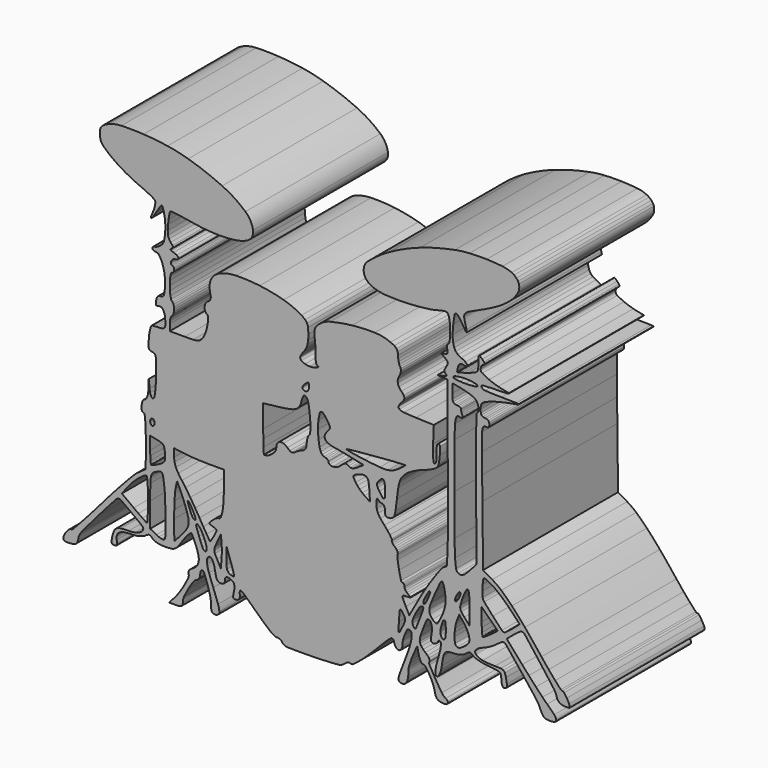
from build123d import *

# Parameters (mm, degrees)
F1_DEPTH = 40


# Not quite as in the source:
# - ends of sketch curves that miss each other by under 0.0002 mm in the source are joined


with BuildPart() as f1:
    # F0 (on Front) → F1 (new body)
    with BuildSketch(Plane.XZ):
        with BuildLine():
            ThreePointArc((22.5855627834, 47.413232074), (20.838311355, 47.2544371655), (19.1050182403, 46.9827786383))
            ThreePointArc((19.1050182403, 46.9827786383), (14.9541308222, 46.0336828181), (10.8845297381, 44.7810870798))
            ThreePointArc((10.8845297381, 44.7810870798), (7.1611396159, 43.2952502008), (3.5834516552, 41.4865229823))
            ThreePointArc((3.5834516552, 41.4865229823), (0.931594568, 39.8150231711), (-1.5396414122, 37.8864873457))
            ThreePointArc((-1.5396414122, 37.8864873457), (-2.409722972, 36.5190183908), (-2.3837905546, 34.8984195056))
            ThreePointArc((-2.3837905546, 34.8984195056), (-2.0345918587, 34.1815507438), (-1.4938622174, 33.5955030419))
            ThreePointArc((-1.4938622174, 33.5955030419), (-0.7215124531, 33.083165563), (0.1329369685, 32.7240972056))
            ThreePointArc((0.1329369685, 32.7240972056), (1.3862342256, 32.410799102), (2.6676761766, 32.2470426258))
            ThreePointArc((2.6676761766, 32.2470426258), (4.5307505685, 32.1580005163), (6.3959068704, 32.1450894058))
            ThreePointArc((6.3959068704, 32.1450894058), (7.4901601107, 32.172352345), (8.583505781, 32.2245890157))
            ThreePointArc((8.583505781, 32.2245890157), (9.7399921819, 32.304245036), (10.8947335822, 32.406118303))
            ThreePointArc((10.8947335822, 32.406118303), (11.9477206197, 32.5195782882), (12.9983003027, 32.6535081213))
            ThreePointArc((12.9983003027, 32.6535081213), (13.7396232073, 32.7753300523), (14.473500833, 32.9360281215))
            ThreePointArc((14.473500833, 32.9360281215), (15.4084096754, 33.1608054649), (16.3459339587, 33.3744116868))
            ThreePointArc((16.3459339587, 33.3744116868), (16.6902812097, 33.421376515), (17.037665783, 33.4111457365))
            ThreePointArc((17.037665783, 33.4111457365), (17.254721153, 33.3362724595), (17.4191366788, 33.1760020487))
            ThreePointArc((17.4191366788, 33.1760020487), (17.5772065355, 32.8859802525), (17.6877261433, 32.5747180729))
            ThreePointArc((17.6877261433, 32.5747180729), (17.8463842657, 31.8439496014), (17.9335637062, 31.1012554051))
            ThreePointArc((17.9335637062, 31.1012554051), (17.9753376926, 30.1557857654), (17.9712811718, 29.2094024038))
            ThreePointArc((17.9712811718, 29.2094024038), (17.9304691922, 28.3134338496), (17.859201745, 27.4193722099))
            ThreePointArc((17.859201745, 27.4193722099), (17.755123357, 27.1122365387), (17.5254353344, 26.8833085916))
            ThreePointArc((17.5254353344, 26.8833085916), (17.4314040703, 26.8030170519), (17.3659642445, 26.6981064473))
            ThreePointArc((17.3659642445, 26.6981064473), (17.3100685742, 26.5403813591), (17.2747498811, 26.3768145276))
            ThreePointArc((17.2747498811, 26.3768145276), (17.2561268683, 26.1787902136), (17.2593312005, 25.9799179259))
            ThreePointArc((17.2593312005, 25.9799179259), (17.2839869462, 25.7705687199), (17.3278463121, 25.5643859171))
            ThreePointArc((17.3278463121, 25.5643859171), (17.3785068266, 25.3218265538), (17.4047581348, 25.0754276916))
            ThreePointArc((17.4047581348, 25.0754276916), (17.3877115077, 24.9120316786), (17.3200675195, 24.7623214484))
            ThreePointArc((17.3200675195, 24.7623214484), (17.2127707366, 24.6499833419), (17.0730677387, 24.5820456973))
            ThreePointArc((17.0730677387, 24.5820456973), (16.8562135851, 24.5357490461), (16.6352079828, 24.5177039327))
            ThreePointArc((16.6352079828, 24.5177039327), (16.3388690176, 24.5088380536), (16.0428565095, 24.4923461943))
            ThreePointArc((16.0428565095, 24.4923461943), (15.9793217119, 24.4607223045), (15.9568402788, 24.3934070856))
            ThreePointArc((15.9568402788, 24.3934070856), (15.9820743926, 24.3052062832), (16.0407515706, 24.2346859358))
            ThreePointArc((16.0407515706, 24.2346859358), (16.3645465448, 23.981473862), (16.6910892894, 23.7318153427))
            ThreePointArc((16.6910892894, 23.7318153427), (16.9656007923, 23.5092414366), (17.2243510615, 23.2685258123))
            ThreePointArc((17.2243510615, 23.2685258123), (17.3469733273, 23.1023683036), (17.4143472426, 22.907162555))
            ThreePointArc((17.4143472426, 22.907162555), (17.4204588766, 22.7003458474), (17.3647468612, 22.5010805569))
            ThreePointArc((17.3647468612, 22.5010805569), (17.2079703527, 22.1825245163), (17.0301359102, 21.8752270522))
            ThreePointArc((17.0301359102, 21.8752270522), (16.861314254, 21.5896464658), (16.7065996828, 21.2961836547))
            ThreePointArc((16.7065996828, 21.2961836547), (16.6405119272, 21.1151323378), (16.6158407273, 20.9239818892))
            ThreePointArc((16.6158407273, 20.9239818892), (16.6394961564, 20.7741676471), (16.7128624529, 20.6414224663))
            ThreePointArc((16.7128624529, 20.6414224663), (16.8475493268, 20.5007311677), (17.0039907306, 20.3847110775))
            ThreePointArc((17.0039907306, 20.3847110775), (17.0969595656, 20.3040396735), (17.1595965121, 20.1980789501))
            ThreePointArc((17.1595965121, 20.1980789501), (17.1638405759, 20.1040258639), (17.1098884529, 20.0268692428))
            ThreePointArc((17.1098884529, 20.0268692428), (16.9551804088, 19.9359465712), (16.7853089932, 19.8781087156))
            ThreePointArc((16.7853089932, 19.8781087156), (16.4686193309, 19.8116913607), (16.1495416892, 19.7579040671))
            ThreePointArc((16.1495416892, 19.7579040671), (15.6299324623, 19.6804888209), (15.1104418379, 19.6022816586))
            ThreePointArc((15.1104418379, 19.6022816586), (15.0718025233, 19.5865957042), (15.0444853674, 19.5550866024))
            ThreePointArc((15.0444853674, 19.5550866024), (15.0449962509, 19.5270423122), (15.0687833828, 19.5121787843))
            ThreePointArc((15.0687833828, 19.5121787843), (15.5311109655, 19.4842338306), (15.9934985225, 19.4572994446))
            Line((15.9934985225, 19.4572994446), (17.3446587822, 19.3800757262))
            Line((17.3446587822, 19.3800757262), (17.4326234659, -0.141702862))
            ThreePointArc((17.4326234659, -0.141702862), (17.4510166929, -5.5900176021), (17.4570856374, -11.0383600094))
            ThreePointArc((17.4570856374, -11.0383600094), (17.435271916, -13.6306275743), (17.3699248011, -16.2221631641))
            ThreePointArc((17.3699248011, -16.2221631641), (17.3026513662, -17.791308934), (17.2063968677, -19.3589438546))
            ThreePointArc((17.2063968677, -19.3589438546), (17.0729711451, -19.7199539257), (16.7665447427, -19.9528347384))
            ThreePointArc((16.7665447427, -19.9528347384), (16.2854666112, -20.2194728464), (15.8965722812, -20.6084372486))
            ThreePointArc((15.8965722812, -20.6084372486), (14.9704522339, -21.8627921017), (14.068652633, -23.1347441086))
            ThreePointArc((14.068652633, -23.1347441086), (13.0446552317, -24.6527492317), (12.0624827011, -26.1981447693))
            ThreePointArc((12.0624827011, -26.1981447693), (11.0669381233, -27.8555938436), (10.1101091094, -29.5356904718))
            Line((10.1101091094, -29.5356904718), (8.2955872726, -32.8095377899))
            Line((8.2955872726, -32.8095377899), (7.4745978176, -31.2219188403))
            ThreePointArc((7.4745978176, -31.2219188403), (7.1309562023, -30.5431965314), (6.7989958335, -29.8586851425))
            ThreePointArc((6.7989958335, -29.8586851425), (6.7276794045, -29.6227388155), (6.7290046962, -29.3762535475))
            ThreePointArc((6.7290046962, -29.3762535475), (6.8125955794, -29.2109115345), (6.9772545718, -29.1259835389))
            ThreePointArc((6.9772545718, -29.1259835389), (7.3938766124, -29.073387928), (7.8132622627, -29.0520359027))
            ThreePointArc((7.8132622627, -29.0520359027), (8.1618320921, -29.0449153783), (8.5102702189, -29.0329781152))
            ThreePointArc((8.5102702189, -29.0329781152), (8.5826393107, -29.0096023196), (8.6325461253, -28.9522173888))
            ThreePointArc((8.6325461253, -28.9522173888), (8.6380552746, -28.8852776894), (8.597796816, -28.8315139253))
            ThreePointArc((8.597796816, -28.8315139253), (8.3359113452, -28.6687515197), (8.0709632508, -28.5110235639))
            ThreePointArc((8.0709632508, -28.5110235639), (7.8912950293, -28.3924622933), (7.7259716658, -28.2546013707))
            ThreePointArc((7.7259716658, -28.2546013707), (7.5714632896, -28.0949432601), (7.4339589644, -27.9204264762))
            ThreePointArc((7.4339589644, -27.9204264762), (7.3246767812, -27.7470154176), (7.2347838431, -27.5628056092))
            ThreePointArc((7.2347838431, -27.5628056092), (7.1856187021, -27.4037968822), (7.1690098094, -27.2381915297))
            ThreePointArc((7.1690098094, -27.2381915297), (7.1604862099, -27.094250706), (7.1350345469, -26.9523217613))
            ThreePointArc((7.1350345469, -26.9523217613), (7.094378157, -26.8273806), (7.0348013307, -26.7102744972))
            ThreePointArc((7.0348013307, -26.7102744972), (6.9684298559, -26.6220447338), (6.8863961462, -26.5481520852))
            ThreePointArc((6.8863961462, -26.5481520852), (6.8038756684, -26.5054325579), (6.7121286476, -26.4906989099))
            ThreePointArc((6.7121286476, -26.4906989099), (6.4787188484, -26.4102104727), (6.3445313199, -26.2029612746))
            ThreePointArc((6.3445313199, -26.2029612746), (6.103435635, -25.1840812114), (5.8831241962, -24.1605058173))
            ThreePointArc((5.8831241962, -24.1605058173), (5.6946672822, -23.1477905074), (5.5424605654, -22.1289964061))
            ThreePointArc((5.5424605654, -22.1289964061), (5.5089390025, -21.5147979372), (5.5687271496, -20.902597913))
            ThreePointArc((5.5687271496, -20.902597913), (5.578423849, -20.74677138), (5.5535289679, -20.5926409734))
            ThreePointArc((5.5535289679, -20.5926409734), (5.4905602352, -20.4085151456), (5.4066187078, -20.2329554713))
            ThreePointArc((5.4066187078, -20.2329554713), (5.2928597622, -20.0506453131), (5.1602382305, -19.8815605965))
            ThreePointArc((5.1602382305, -19.8815605965), (5.0114593609, -19.7293273634), (4.8468227517, -19.594401915))
            ThreePointArc((4.8468227517, -19.594401915), (4.6851754301, -19.4649733742), (4.5354665598, -19.3219039808))
            ThreePointArc((4.5354665598, -19.3219039808), (4.4076574357, -19.1739042959), (4.2958919372, -19.0134438322))
            ThreePointArc((4.2958919372, -19.0134438322), (4.2177449184, -18.8691583912), (4.1574465466, -18.7165499239))
            ThreePointArc((4.1574465466, -18.7165499239), (4.1381957535, -18.5995945627), (4.1550965782, -18.4822766081))
            ThreePointArc((4.1550965782, -18.4822766081), (4.1686575748, -18.3304502786), (4.1199693666, -18.1860045684))
            ThreePointArc((4.1199693666, -18.1860045684), (3.9154182615, -17.8525094325), (3.6990102047, -17.5265834863))
            ThreePointArc((3.6990102047, -17.5265834863), (3.4143705001, -17.1324442543), (3.1131736774, -16.7508083503))
            ThreePointArc((3.1131736774, -16.7508083503), (2.7577406287, -16.332511913), (2.3900385904, -15.9249585102))
            ThreePointArc((2.3900385904, -15.9249585102), (1.905837696, -15.3813863741), (1.4451115919, -14.8177795555))
            ThreePointArc((1.4451115919, -14.8177795555), (1.1401026258, -14.3824373576), (0.8828247542, -13.9172907348))
            ThreePointArc((0.8828247542, -13.9172907348), (0.7099097828, -13.492036019), (0.5945378362, -13.0477045349))
            ThreePointArc((0.5945378362, -13.0477045349), (0.5273760601, -12.5557357887), (0.5119361562, -12.0594439645))
            ThreePointArc((0.5119361562, -12.0594439645), (0.5233859133, -11.7325586833), (0.5438668183, -11.4061147949))
            ThreePointArc((0.5438668183, -11.4061147949), (0.5701276355, -11.1888338042), (0.6152980427, -10.9746836202))
            ThreePointArc((0.6152980427, -10.9746836202), (0.6499391585, -10.9068935351), (0.7102232007, -10.860403312))
            ThreePointArc((0.7102232007, -10.860403312), (0.7686369954, -10.8586311351), (0.8101255809, -10.8997894107))
            ThreePointArc((0.8101255809, -10.8997894107), (0.8762713436, -11.0296930933), (0.9640131557, -11.1461045215))
            ThreePointArc((0.9640131557, -11.1461045215), (1.0793014622, -11.2584148105), (1.2082055562, -11.3547928509))
            ThreePointArc((1.2082055562, -11.3547928509), (1.3503993689, -11.4348056105), (1.5016813244, -11.4959192834))
            ThreePointArc((1.5016813244, -11.4959192834), (1.6490338113, -11.5319341001), (1.8002397134, -11.544042006))
            ThreePointArc((1.8002397134, -11.544042006), (1.9557390785, -11.5687390457), (2.0959345495, -11.6403995383))
            ThreePointArc((2.0959345495, -11.6403995383), (2.2278149972, -11.7606387268), (2.3305031665, -11.9066013009))
            ThreePointArc((2.3305031665, -11.9066013009), (2.4226830251, -12.1110952412), (2.4809468446, -12.327705996))
            ThreePointArc((2.4809468446, -12.327705996), (2.5180051226, -12.5969217425), (2.5303921496, -12.8683936334))
            ThreePointArc((2.5303921496, -12.8683936334), (2.5426716797, -13.2103475898), (2.5794470864, -13.5505399833))
            ThreePointArc((2.5794470864, -13.5505399833), (2.6392239923, -13.7410591214), (2.7560452438, -13.9029962631))
            ThreePointArc((2.7560452438, -13.9029962631), (2.910516279, -14.0093476892), (3.0927678481, -14.0535774272))
            ThreePointArc((3.0927678481, -14.0535774272), (3.3920354994, -14.0555121256), (3.6900465721, -14.0280481015))
            ThreePointArc((3.6900465721, -14.0280481015), (4.0329701282, -13.9316889365), (4.3385581736, -13.7486654952))
            ThreePointArc((4.3385581736, -13.7486654952), (4.581673753, -13.4935172443), (4.7466393046, -13.1820815702))
            ThreePointArc((4.7466393046, -13.1820815702), (4.9174832655, -12.6248907305), (5.028946213, -12.0528545943))
            ThreePointArc((5.028946213, -12.0528545943), (5.2048346337, -10.7474060925), (5.3651031607, -9.4399480527))
            ThreePointArc((5.3651031607, -9.4399480527), (5.5228975317, -8.1848361994), (5.7034370224, -6.9327937379))
            ThreePointArc((5.7034370224, -6.9327937379), (5.8430839169, -6.2325037789), (6.0444908467, -5.5474179963))
            ThreePointArc((6.0444908467, -5.5474179963), (6.2582236718, -5.0453452469), (6.5417759018, -4.5791297384))
            ThreePointArc((6.5417759018, -4.5791297384), (6.9198986213, -4.1022771476), (7.3455006038, -3.6672735584))
            ThreePointArc((7.3455006038, -3.6672735584), (7.7073201101, -3.361391607), (8.0937930208, -3.0873189527))
            ThreePointArc((8.0937930208, -3.0873189527), (8.6195480737, -2.7613922826), (9.1575671256, -2.456134893))
            ThreePointArc((9.1575671256, -2.456134893), (9.7414437367, -2.153957086), (10.3364217768, -1.8742707291))
            ThreePointArc((10.3364217768, -1.8742707291), (10.8912921206, -1.6426572209), (11.4570108971, -1.4389707637))
            ThreePointArc((11.4570108971, -1.4389707637), (11.9902683102, -1.2538054085), (12.5183218205, -1.0542830773))
            ThreePointArc((12.5183218205, -1.0542830773), (13.0218260938, -0.8473906587), (13.5188610041, -0.6254056778))
            ThreePointArc((13.5188610041, -0.6254056778), (13.935458263, -0.4243533048), (14.346044417, -0.2112938327))
            ThreePointArc((14.346044417, -0.2112938327), (14.5641218603, -0.0726692529), (14.7596932024, 0.0962283548))
            ThreePointArc((14.7596932024, 0.0962283548), (15.0823321446, 0.5310454085), (15.2650942046, 1.0407117285))
            ThreePointArc((15.2650942046, 1.0407117285), (15.4255761512, 1.9904561608), (15.5290368335, 2.9480911842))
            ThreePointArc((15.5290368335, 2.9480911842), (15.5765491906, 3.8738292099), (15.5750372126, 4.8007844628))
            ThreePointArc((15.5750372126, 4.8007844628), (15.4487556432, 5.0883667118), (15.1577402236, 5.2065217656))
            ThreePointArc((15.1577402236, 5.2065217656), (15.0403132135, 5.1693284201), (14.9657117424, 5.0713127675))
            ThreePointArc((14.9657117424, 5.0713127675), (14.8874351727, 4.8200267317), (14.8304471072, 4.5630748835))
            ThreePointArc((14.8304471072, 4.5630748835), (14.7807259994, 4.2107113373), (14.7566297499, 3.8556738365))
            ThreePointArc((14.7566297499, 3.8556738365), (14.7526733892, 3.4357504423), (14.7673061628, 3.0160634225))
            ThreePointArc((14.7673061628, 3.0160634225), (14.7833208276, 2.5722972337), (14.7807635621, 2.1282495386))
            ThreePointArc((14.7807635621, 2.1282495386), (14.7567110708, 1.7786319326), (14.7033996573, 1.4322666622))
            ThreePointArc((14.7033996573, 1.4322666622), (14.6421374104, 1.194985289), (14.5538553682, 0.9663769295))
            ThreePointArc((14.5538553682, 0.9663769295), (14.4652705735, 0.86384328), (14.3352772343, 0.8256050869))
            ThreePointArc((14.3352772343, 0.8256050869), (14.1810714611, 0.8796774481), (14.094403552, 1.0182123329))
            ThreePointArc((14.094403552, 1.0182123329), (14.0155587957, 1.4268512851), (13.9623292459, 1.8396089654))
            ThreePointArc((13.9623292459, 1.8396089654), (13.9181443841, 2.4555664163), (13.9053774341, 3.0729746285))
            ThreePointArc((13.9053774341, 3.0729746285), (13.917700404, 3.9466629522), (13.9462909804, 4.819970295))
            Line((13.9462909804, 4.819970295), (14.1143017355, 8.814335501))
            Line((14.1143017355, 8.814335501), (9.8685528291, 8.9640303931))
            ThreePointArc((9.8685528291, 8.9640303931), (8.4711170875, 9.0285407922), (7.0754174427, 9.1234657526))
            ThreePointArc((7.0754174427, 9.1234657526), (6.5047488643, 9.2325937096), (5.971719715, 9.463789395))
            ThreePointArc((5.971719715, 9.463789395), (5.7644111897, 9.7170634313), (5.7791358877, 10.0440308759))
            ThreePointArc((5.7791358877, 10.0440308759), (6.0449573808, 10.5257921453), (6.3959070228, 10.9495719713))
            ThreePointArc((6.3959070228, 10.9495719713), (6.6893943888, 11.2706826931), (6.9528914338, 11.6168275029))
            ThreePointArc((6.9528914338, 11.6168275029), (7.0796774614, 11.8736836323), (7.1264672969, 12.1562796444))
            ThreePointArc((7.1264672969, 12.1562796444), (7.0885463431, 12.4356101418), (6.9688544918, 12.6908303434))
            ThreePointArc((6.9688544918, 12.6908303434), (6.7183508317, 13.027924791), (6.4362097122, 13.3390214544))
            ThreePointArc((6.4362097122, 13.3390214544), (6.1177970316, 13.6994753041), (5.8462912495, 14.0964617446))
            ThreePointArc((5.8462912495, 14.0964617446), (5.6734389736, 14.4660523259), (5.577883489, 14.8627187394))
            ThreePointArc((5.577883489, 14.8627187394), (5.5632009124, 15.2719357154), (5.6301026733, 15.67591374))
            ThreePointArc((5.6301026733, 15.67591374), (5.78486293, 16.1355775124), (5.9941093937, 16.5731360506))
            ThreePointArc((5.9941093937, 16.5731360506), (6.1135622172, 16.8148749264), (6.2094065094, 17.0669077734))
            ThreePointArc((6.2094065094, 17.0669077734), (6.2709173684, 17.3050468866), (6.3020890772, 17.5490184937))
            ThreePointArc((6.3020890772, 17.5490184937), (6.3007281383, 17.772440103), (6.2680629311, 17.9934650826))
            ThreePointArc((6.2680629311, 17.9934650826), (6.2057810888, 18.1921220459), (6.1101358976, 18.3770425855))
            ThreePointArc((6.1101358976, 18.3770425855), (6.0071832681, 18.5646054214), (5.9282574108, 18.7634766503))
            ThreePointArc((5.9282574108, 18.7634766503), (5.8444642364, 19.0435715077), (5.7747874174, 19.3275073508))
            ThreePointArc((5.7747874174, 19.3275073508), (5.7139146279, 19.6417784282), (5.6683769879, 19.9586350678))
            ThreePointArc((5.6683769879, 19.9586350678), (5.6409562872, 20.2618000142), (5.630696377, 20.5660295577))
            ThreePointArc((5.630696377, 20.5660295577), (5.6064592346, 20.949098712), (5.5382612956, 21.326826712))
            ThreePointArc((5.5382612956, 21.326826712), (5.433781276, 21.6140338181), (5.2678282518, 21.8706729049))
            ThreePointArc((5.2678282518, 21.8706729049), (5.0270979345, 22.1146407242), (4.7457335222, 22.3103584324))
            ThreePointArc((4.7457335222, 22.3103584324), (4.2972772156, 22.5470628818), (3.8354512505, 22.756487896))
            ThreePointArc((3.8354512505, 22.756487896), (2.0266593536, 23.3211162055), (0.1445583286, 23.5407272066))
            ThreePointArc((0.1445583286, 23.5407272066), (-2.5564786213, 23.5122270236), (-5.2495458352, 23.3029381695))
            ThreePointArc((-5.2495458352, 23.3029381695), (-7.8654582115, 22.9252820515), (-10.4515173933, 22.3794619459))
            ThreePointArc((-10.4515173933, 22.3794619459), (-11.9606291002, 21.7962297097), (-13.2719958796, 20.8486563762))
            ThreePointArc((-13.2719958796, 20.8486563762), (-13.5684522992, 20.5415198905), (-13.8335008335, 20.206902954))
            ThreePointArc((-13.8335008335, 20.206902954), (-14.0085854137, 19.9083112369), (-14.1269504774, 19.5830400208))
            ThreePointArc((-14.1269504774, 19.5830400208), (-14.1986652442, 19.1991580412), (-14.21326378, 18.8089077838))
            ThreePointArc((-14.21326378, 18.8089077838), (-14.1785301053, 18.2297075636), (-14.1164603302, 17.6527962515))
            ThreePointArc((-14.1164603302, 17.6527962515), (-14.0597911712, 17.1828662172), (-14.0132912141, 16.7118212241))
            ThreePointArc((-14.0132912141, 16.7118212241), (-13.970793504, 16.1815136874), (-13.9363851638, 15.6506199094))
            ThreePointArc((-13.9363851638, 15.6506199094), (-13.9112412576, 15.1420498893), (-13.8939298835, 14.633153045))
            ThreePointArc((-13.8939298835, 14.633153045), (-13.8898505477, 14.2362922633), (-13.8984933264, 13.8395046343))
            ThreePointArc((-13.8984933264, 13.8395046343), (-13.9007157041, 13.4955499196), (-13.8813857906, 13.1521316135))
            ThreePointArc((-13.8813857906, 13.1521316135), (-13.8408219113, 12.8783500294), (-13.7680305527, 12.6113234235))
            ThreePointArc((-13.7680305527, 12.6113234235), (-13.6868547985, 12.4252769811), (-13.5751138797, 12.2558168367))
            ThreePointArc((-13.5751138797, 12.2558168367), (-13.4608526722, 12.160794067), (-13.3179089303, 12.1201486682))
            ThreePointArc((-13.3179089303, 12.1201486682), (-13.2719908793, 12.0992040186), (-13.251210373, 12.0532116197))
            ThreePointArc((-13.251210373, 12.0532116197), (-13.2631456126, 11.998011848), (-13.3024220523, 11.9574307053))
            ThreePointArc((-13.3024220523, 11.9574307053), (-13.4646365424, 11.8732828024), (-13.6337772418, 11.8041031332))
            ThreePointArc((-13.6337772418, 11.8041031332), (-13.9004624186, 11.7127558908), (-14.1694489437, 11.6284258781))
            ThreePointArc((-14.1694489437, 11.6284258781), (-14.7241886613, 11.5059776037), (-15.2908774512, 11.4660578922))
            ThreePointArc((-15.2908774512, 11.4660578922), (-15.8646965987, 11.5085111388), (-16.4268017786, 11.6314276231))
            ThreePointArc((-16.4268017786, 11.6314276231), (-16.8699918348, 11.8044501986), (-17.2769270403, 12.0509415452))
            ThreePointArc((-17.2769270403, 12.0509415452), (-17.4927413131, 12.3045923855), (-17.5702843764, 12.628477527))
            ThreePointArc((-17.5702843764, 12.628477527), (-17.5561788517, 12.750431112), (-17.514607125, 12.8659448958))
            ThreePointArc((-17.514607125, 12.8659448958), (-17.4014292275, 13.0843785329), (-17.2807001392, 13.2987309924))
            ThreePointArc((-17.2807001392, 13.2987309924), (-17.1260041669, 13.5515154555), (-16.9619220252, 13.7983106748))
            ThreePointArc((-16.9619220252, 13.7983106748), (-16.7770913253, 14.0567848423), (-16.5844661705, 14.3095037178))
            ThreePointArc((-16.5844661705, 14.3095037178), (-16.3449360982, 14.6527068197), (-16.1461370336, 15.021002823))
            ThreePointArc((-16.1461370336, 15.021002823), (-15.9763630261, 15.4334438668), (-15.8462944795, 15.8600736734))
            ThreePointArc((-15.8462944795, 15.8600736734), (-15.7418908027, 16.3549892795), (-15.6781080401, 16.8567594894))
            ThreePointArc((-15.6781080401, 16.8567594894), (-15.6421645146, 17.4501379993), (-15.6361670934, 18.0445738894))
            ThreePointArc((-15.6361670934, 18.0445738894), (-15.6609502154, 18.7569656686), (-15.7137165332, 19.4678327307))
            ThreePointArc((-15.7137165332, 19.4678327307), (-15.7890147, 19.8809508504), (-15.9343296898, 20.2749304322))
            ThreePointArc((-15.9343296898, 20.2749304322), (-16.1309096291, 20.5980831056), (-16.3914260047, 20.8723139671))
            ThreePointArc((-16.3914260047, 20.8723139671), (-16.8167451796, 21.2067956356), (-17.2662376591, 21.5080112965))
            ThreePointArc((-17.2662376591, 21.5080112965), (-19.3141487409, 22.5780619603), (-21.4927185143, 23.3479854415))
            ThreePointArc((-21.4927185143, 23.3479854415), (-24.3068204743, 24.0134306931), (-27.162064305, 24.4712188139))
            ThreePointArc((-27.162064305, 24.4712188139), (-29.9598621032, 24.7121381713), (-32.7677776287, 24.7485389021))
            ThreePointArc((-32.7677776287, 24.7485389021), (-34.7709565996, 24.5099384773), (-36.6929677384, 23.8971340021))
            ThreePointArc((-36.6929677384, 23.8971340021), (-37.351503222, 23.5457515422), (-37.9397617478, 23.0863056466))
            ThreePointArc((-37.9397617478, 23.0863056466), (-38.4013777708, 22.5573981422), (-38.7441838693, 21.9447673937))
            ThreePointArc((-38.7441838693, 21.9447673937), (-38.9674034192, 21.2456013955), (-39.0510413792, 20.5164478967))
            ThreePointArc((-39.0510413792, 20.5164478967), (-39.0085427533, 19.6895656335), (-38.8540958964, 18.8761244765))
            ThreePointArc((-38.8540958964, 18.8761244765), (-38.7982002206, 18.6048929825), (-38.7710616833, 18.3292948203))
            ThreePointArc((-38.7710616833, 18.3292948203), (-38.7814999989, 18.0996533991), (-38.8333483355, 17.8756982644))
            ThreePointArc((-38.8333483355, 17.8756982644), (-38.9198519348, 17.6826505179), (-39.0439195053, 17.5113100994))
            ThreePointArc((-39.0439195053, 17.5113100994), (-39.2090472468, 17.3548144772), (-39.3977099509, 17.2276750335))
            ThreePointArc((-39.3977099509, 17.2276750335), (-39.7121908025, 16.9899894514), (-39.9506259348, 16.6760764796))
            ThreePointArc((-39.9506259348, 16.6760764796), (-40.1272473066, 16.2733241226), (-40.2209256782, 15.8436394528))
            ThreePointArc((-40.2209256782, 15.8436394528), (-40.2248191665, 15.4260102417), (-40.1407299143, 15.016915702))
            ThreePointArc((-40.1407299143, 15.016915702), (-39.9773325624, 14.707505272), (-39.7167539668, 14.4739838261))
            ThreePointArc((-39.7167539668, 14.4739838261), (-39.4640422908, 14.2050333324), (-39.3804836597, 13.8455678179))
            ThreePointArc((-39.3804836597, 13.8455678179), (-39.4354332256, 13.054680451), (-39.545281855, 12.2695336289))
            ThreePointArc((-39.545281855, 12.2695336289), (-39.7320230837, 11.4034310034), (-39.984891423, 10.5542763161))
            ThreePointArc((-39.984891423, 10.5542763161), (-40.2716319188, 9.8570868366), (-40.6427047241, 9.2008869841))
            ThreePointArc((-40.6427047241, 9.2008869841), (-40.8973133371, 8.8699067363), (-41.2007262319, 8.583002415))
            ThreePointArc((-41.2007262319, 8.583002415), (-41.5200818486, 8.3761490269), (-41.8752276605, 8.2395921397))
            ThreePointArc((-41.8752276605, 8.2395921397), (-42.3953860332, 8.1303331441), (-42.9245165019, 8.0801017118))
            ThreePointArc((-42.9245165019, 8.0801017118), (-43.9350035239, 8.0509504573), (-44.9458642374, 8.0412325577))
            Line((-44.9458642374, 8.0412325577), (-48.4944021086, 8.0412325577))
            Line((-48.4944021086, 8.0412325577), (-48.4944021086, 9.5570209667))
            ThreePointArc((-48.4944021086, 9.5570209667), (-48.4849078895, 9.8594186858), (-48.4564623086, 10.1606252091))
            ThreePointArc((-48.4564623086, 10.1606252091), (-48.4101320146, 10.4429760543), (-48.3430025881, 10.7211165459))
            ThreePointArc((-48.3430025881, 10.7211165459), (-48.2693696557, 10.9476806614), (-48.1777272471, 11.1675778614))
            ThreePointArc((-48.1777272471, 11.1675778614), (-48.0947599131, 11.2940230199), (-47.9790001703, 11.3913453508))
            ThreePointArc((-47.9790001703, 11.3913453508), (-47.8665846217, 11.4825187034), (-47.7808860836, 11.5991617157))
            ThreePointArc((-47.7808860836, 11.5991617157), (-47.6892451416, 11.7842316771), (-47.6149974325, 11.9769393261))
            ThreePointArc((-47.6149974325, 11.9769393261), (-47.5485326471, 12.2082269228), (-47.5016708696, 12.4442682181))
            ThreePointArc((-47.5016708696, 12.4442682181), (-47.4731304536, 12.6901761631), (-47.4635981841, 12.9375511987))
            ThreePointArc((-47.4635981841, 12.9375511987), (-47.4731304536, 13.1849262342), (-47.5016708881, 13.4308341763))
            ThreePointArc((-47.5016708881, 13.4308341763), (-47.5485326471, 13.6668754745), (-47.6149974698, 13.8981630588))
            ThreePointArc((-47.6149974698, 13.8981630588), (-47.6892454673, 14.0908708292), (-47.7808860718, 14.2759412035))
            ThreePointArc((-47.7808860718, 14.2759412035), (-47.8665845943, 14.3925839996), (-47.9790002135, 14.4837569766))
            ThreePointArc((-47.9790002135, 14.4837569766), (-48.1063622831, 14.6013071101), (-48.1804807592, 14.757977297))
            ThreePointArc((-48.1804807592, 14.757977297), (-48.2701211952, 15.1434726269), (-48.3430026469, 15.5324846506))
            ThreePointArc((-48.3430026469, 15.5324846506), (-48.4115301584, 16.0195082424), (-48.4568278402, 16.5092388941))
            ThreePointArc((-48.4568278402, 16.5092388941), (-48.4850057367, 17.0575910624), (-48.4944021085, 17.6065863361))
            ThreePointArc((-48.4944021085, 17.6065863361), (-48.4851024539, 18.1443955715), (-48.4572143243, 18.6815617558))
            ThreePointArc((-48.4572143243, 18.6815617558), (-48.4128576171, 19.1359482672), (-48.3430025104, 19.5871188293))
            ThreePointArc((-48.3430025104, 19.5871188293), (-48.2709884762, 19.9262918867), (-48.1804678441, 20.2610013244))
            ThreePointArc((-48.1804678441, 20.2610013244), (-48.104551549, 20.3693005681), (-47.9790001463, 20.4108796506))
            ThreePointArc((-47.9790001463, 20.4108796506), (-47.8763110396, 20.4260976721), (-47.7824490186, 20.470443606))
            ThreePointArc((-47.7824490186, 20.470443606), (-47.6904391223, 20.5459311078), (-47.614997484, 20.6379786225))
            ThreePointArc((-47.614997484, 20.6379786225), (-47.5482252879, 20.7585475344), (-47.5020957387, 20.8884222782))
            ThreePointArc((-47.5020957387, 20.8884222782), (-47.4732629283, 21.0349540859), (-47.4635981841, 21.1839825939))
            ThreePointArc((-47.4635981841, 21.1839825939), (-47.4729416424, 21.3329498417), (-47.5008256917, 21.479582106))
            ThreePointArc((-47.5008256917, 21.479582106), (-47.5454091145, 21.6092093167), (-47.6102454218, 21.729986601))
            ThreePointArc((-47.6102454218, 21.729986601), (-47.683114242, 21.8217333627), (-47.7724319632, 21.897560036))
            ThreePointArc((-47.7724319632, 21.897560036), (-47.8630839872, 21.9418572553), (-47.9628242558, 21.9570855372))
            ThreePointArc((-47.9628242558, 21.9570855372), (-48.0512620779, 21.973405321), (-48.1280503798, 22.0202149399))
            ThreePointArc((-48.1280503798, 22.0202149399), (-48.1902217812, 22.0948245324), (-48.2282563496, 22.18418464))
            ThreePointArc((-48.2282563496, 22.18418464), (-48.2478614923, 22.3084618575), (-48.2424394668, 22.4341590961))
            ThreePointArc((-48.2424394668, 22.4341590961), (-48.2121908741, 22.5843289929), (-48.1653830389, 22.7301885352))
            ThreePointArc((-48.1653830389, 22.7301885352), (-48.0928103081, 22.8841591905), (-47.9983126486, 23.0257358459))
            ThreePointArc((-47.9983126486, 23.0257358459), (-47.8796961457, 23.1591167475), (-47.7449606124, 23.2761922485))
            ThreePointArc((-47.7449606124, 23.2761922485), (-47.6018407348, 23.3708522111), (-47.4473929651, 23.4456165205))
            ThreePointArc((-47.4473929651, 23.4456165205), (-47.3018513199, 23.4887389722), (-47.1507548625, 23.5032914238))
            ThreePointArc((-47.1507548625, 23.5032914238), (-46.8649275839, 23.5395838996), (-46.5972404708, 23.6461577542))
            ThreePointArc((-46.5972404708, 23.6461577542), (-46.468956687, 23.7938744191), (-46.4661985772, 23.9894999582))
            ThreePointArc((-46.4661985772, 23.9894999582), (-46.6071851422, 24.2407965472), (-46.8257446095, 24.4285701295))
            ThreePointArc((-46.8257446095, 24.4285701295), (-47.1989582965, 24.6204817011), (-47.5924486774, 24.7663715418))
            ThreePointArc((-47.5924486774, 24.7663715418), (-47.8319239139, 24.8454592106), (-48.0673499332, 24.9358906259))
            ThreePointArc((-48.0673499332, 24.9358906259), (-48.1850170206, 25.0035318549), (-48.2811293669, 25.0993613618))
            ThreePointArc((-48.2811293669, 25.0993613618), (-48.3061685937, 25.1771420387), (-48.2760724171, 25.2531091984))
            ThreePointArc((-48.2760724171, 25.2531091984), (-48.1844392036, 25.335782546), (-48.0763436095, 25.3953382363))
            ThreePointArc((-48.0763436095, 25.3953382363), (-47.9269384017, 25.474763777), (-47.7963493983, 25.5823595214))
            ThreePointArc((-47.7963493983, 25.5823595214), (-47.731223522, 25.6893361214), (-47.7214846615, 25.8141981786))
            ThreePointArc((-47.7214846615, 25.8141981786), (-47.7696304976, 25.9821013949), (-47.8570907202, 26.1332973312))
            ThreePointArc((-47.8570907202, 26.1332973312), (-48.0590634965, 26.3886756005), (-48.2721413974, 26.6348642877))
            ThreePointArc((-48.2721413974, 26.6348642877), (-48.4963604529, 26.92228196), (-48.6763384978, 27.2392851061))
            ThreePointArc((-48.6763384978, 27.2392851061), (-48.8135374623, 27.5872067971), (-48.9025266218, 27.9504615027))
            ThreePointArc((-48.9025266218, 27.9504615027), (-48.9602335746, 28.4150633344), (-48.9722185207, 28.8830818478))
            ThreePointArc((-48.9722185207, 28.8830818478), (-48.9448445595, 29.5425314307), (-48.8936188505, 30.2005580384))
            ThreePointArc((-48.8936188505, 30.2005580384), (-48.8405085844, 30.7089884507), (-48.7789797619, 31.2164688799))
            ThreePointArc((-48.7789797619, 31.2164688799), (-48.7152422111, 31.666418625), (-48.6409247544, 32.1147423524))
            ThreePointArc((-48.6409247544, 32.1147423524), (-48.5720289581, 32.4850098015), (-48.4972795035, 32.8541400397))
            ThreePointArc((-48.4972795035, 32.8541400397), (-48.4560475337, 32.9663508537), (-48.3845611593, 33.0621686319))
            ThreePointArc((-48.3845611593, 33.0621686319), (-48.2788165997, 33.1291216051), (-48.1545965321, 33.1444188916))
            ThreePointArc((-48.1545965321, 33.1444188916), (-47.4668639659, 33.0738801256), (-46.7796850381, 32.9981376711))
            ThreePointArc((-46.7796850381, 32.9981376711), (-45.9683691709, 32.8982850375), (-45.1589581766, 32.7840141723))
            ThreePointArc((-45.1589581766, 32.7840141723), (-44.2210261153, 32.6376080784), (-43.284823662, 32.4805212795))
            ThreePointArc((-43.284823662, 32.4805212795), (-41.2755198064, 32.1790919961), (-39.2544664093, 31.9705140497))
            ThreePointArc((-39.2544664093, 31.9705140497), (-37.381517209, 31.8757911841), (-35.5062345192, 31.8908243598))
            ThreePointArc((-35.5062345192, 31.8908243598), (-33.9082269406, 32.0028858281), (-32.32096843, 32.2192106189))
            ThreePointArc((-32.32096843, 32.2192106189), (-31.1636119925, 32.509121671), (-30.0646720954, 32.9737219815))
            ThreePointArc((-30.0646720954, 32.9737219815), (-28.9948266307, 34.0522777282), (-28.7573888887, 35.5527692215))
            ThreePointArc((-28.7573888887, 35.5527692215), (-29.368409419, 37.3492965731), (-30.5512286179, 38.8331414257))
            ThreePointArc((-30.5512286179, 38.8331414257), (-33.1791796573, 40.8336148132), (-36.0752438077, 42.4213279662))
            ThreePointArc((-36.0752438077, 42.4213279662), (-40.0426194234, 44.0629428969), (-44.1139354808, 45.4265242837))
            ThreePointArc((-44.1139354808, 45.4265242837), (-46.5447362246, 46.0581232609), (-49.0132046453, 46.5211279065))
            ThreePointArc((-49.0132046453, 46.5211279065), (-51.8547174532, 46.8862095502), (-54.7101214166, 47.1189064071))
            ThreePointArc((-54.7101214166, 47.1189064071), (-57.3421531277, 47.214162128), (-59.9758312274, 47.1940569273))
            ThreePointArc((-59.9758312274, 47.1940569273), (-61.5458327083, 47.0026324691), (-63.0545075883, 46.5278186554))
            ThreePointArc((-63.0545075883, 46.5278186554), (-63.6392541816, 46.2517761785), (-64.197243362, 45.9250100627))
            ThreePointArc((-64.197243362, 45.9250100627), (-64.5486484084, 45.6323148087), (-64.8201366498, 45.2642792569))
            ThreePointArc((-64.8201366498, 45.2642792569), (-64.9968421259, 44.8409976351), (-65.0681175172, 44.387884025))
            ThreePointArc((-65.0681175172, 44.387884025), (-65.0633360217, 43.7367772706), (-65.0018134939, 43.0885660115))
            ThreePointArc((-65.0018134939, 43.0885660115), (-64.7448126135, 42.2650179433), (-64.2359015964, 41.5683899761))
            ThreePointArc((-64.2359015964, 41.5683899761), (-63.1328883745, 40.5616129504), (-61.9606116795, 39.6364073023))
            ThreePointArc((-61.9606116795, 39.6364073023), (-60.4353759145, 38.5952934718), (-58.8441152662, 37.658195975))
            ThreePointArc((-58.8441152662, 37.658195975), (-57.041588062, 36.7345236768), (-55.1946275659, 35.9032525206))
            ThreePointArc((-55.1946275659, 35.9032525206), (-54.6362320232, 35.6613426317), (-54.0834007928, 35.406973592))
            ThreePointArc((-54.0834007928, 35.406973592), (-53.5827724033, 35.1608101621), (-53.0895140997, 34.9001926963))
            ThreePointArc((-53.0895140997, 34.9001926963), (-52.687218121, 34.673662515), (-52.2905784985, 34.437368225))
            ThreePointArc((-52.2905784985, 34.437368225), (-52.1339263832, 34.3149520005), (-52.008942766, 34.1603406198))
            ThreePointArc((-52.008942766, 34.1603406198), (-51.940030329, 34.0056814064), (-51.9188371531, 33.8376955462))
            ThreePointArc((-51.9188371531, 33.8376955462), (-51.9346830341, 33.5530583092), (-51.9699894748, 33.2701751011))
            ThreePointArc((-51.9699894748, 33.2701751011), (-52.0354363577, 32.9315609083), (-52.1227266526, 32.5979094823))
            ThreePointArc((-52.1227266526, 32.5979094823), (-52.2366646369, 32.2485055094), (-52.3691946258, 31.9057216135))
            ThreePointArc((-52.3691946258, 31.9057216135), (-52.6723458681, 31.1664983914), (-52.9657117359, 30.4233374954))
            ThreePointArc((-52.9657117359, 30.4233374954), (-52.9466940167, 30.3168202928), (-52.8433896477, 30.2846366108))
            ThreePointArc((-52.8433896477, 30.2846366108), (-52.6664123078, 30.3664837003), (-52.5321734274, 30.5079045626))
            ThreePointArc((-52.5321734274, 30.5079045626), (-52.0221369478, 31.3105817327), (-51.5187978578, 32.1174755361))
            ThreePointArc((-51.5187978578, 32.1174755361), (-51.1196162559, 32.7569232016), (-50.7147031497, 33.3927570224))
            ThreePointArc((-50.7147031497, 33.3927570224), (-50.5960565457, 33.5274540615), (-50.4427962765, 33.6208969289))
            ThreePointArc((-50.4427962765, 33.6208969289), (-50.3191449041, 33.6203058786), (-50.2337276838, 33.5308973227))
            ThreePointArc((-50.2337276838, 33.5308973227), (-50.0992742651, 33.1491133377), (-49.9819317349, 32.7617279189))
            ThreePointArc((-49.9819317349, 32.7617279189), (-49.7430724622, 31.7223513964), (-49.6006996421, 30.6654278926))
            ThreePointArc((-49.6006996421, 30.6654278926), (-49.5446785234, 29.5342320385), (-49.5756608229, 28.4020736881))
            ThreePointArc((-49.5756608229, 28.4020736881), (-49.6797109302, 27.4099833303), (-49.8601929517, 26.4289145693))
            ThreePointArc((-49.8601929517, 26.4289145693), (-50.0832942674, 25.8609521335), (-50.4677420471, 25.3870792227))
            ThreePointArc((-50.4677420471, 25.3870792227), (-50.6656576745, 25.218039767), (-50.8729433614, 25.0606308173))
            ThreePointArc((-50.8729433614, 25.0606308173), (-51.0878146335, 24.916259353), (-51.3107368542, 24.7846597307))
            ThreePointArc((-51.3107368542, 24.7846597307), (-51.5114523311, 24.6817844956), (-51.7180640453, 24.5913321863))
            ThreePointArc((-51.7180640453, 24.5913321863), (-51.8632635048, 24.5485361036), (-52.0139481039, 24.5340953482))
            ThreePointArc((-52.0139481039, 24.5340953482), (-52.1308561346, 24.5242708336), (-52.2444848188, 24.4950727029))
            ThreePointArc((-52.2444848188, 24.4950727029), (-52.3476181972, 24.4479987798), (-52.4402895195, 24.3826958832))
            ThreePointArc((-52.4402895195, 24.3826958832), (-52.514173331, 24.3055717051), (-52.5712311552, 24.2152867848))
            ThreePointArc((-52.5712311552, 24.2152867848), (-52.6058639877, 24.1196892541), (-52.6176178062, 24.018693386))
            ThreePointArc((-52.6176178062, 24.018693386), (-52.6018708923, 23.9157071475), (-52.5560691194, 23.8221318932))
            ThreePointArc((-52.5560691194, 23.8221318932), (-52.4776454256, 23.7299106586), (-52.3827929059, 23.6546908049))
            ThreePointArc((-52.3827929059, 23.6546908049), (-52.2578967266, 23.5877460107), (-52.123872419, 23.5417227626))
            ThreePointArc((-52.123872419, 23.5417227626), (-51.972247235, 23.5129369358), (-51.8182154469, 23.5032914238))
            ThreePointArc((-51.8182154469, 23.5032914238), (-51.3248698022, 23.3763308652), (-50.9540976803, 23.0269930027))
            ThreePointArc((-50.9540976803, 23.0269930027), (-50.5322680477, 22.2646003625), (-50.201356631, 21.4585728102))
            ThreePointArc((-50.201356631, 21.4585728102), (-49.9015565231, 20.4204625211), (-49.7079933736, 19.3574073126))
            ThreePointArc((-49.7079933736, 19.3574073126), (-49.6164477565, 18.2532539972), (-49.6286555692, 17.1453793825))
            ThreePointArc((-49.6286555692, 17.1453793825), (-49.6770738002, 16.4570726724), (-49.7424586152, 15.7701700116))
            ThreePointArc((-49.7424586152, 15.7701700116), (-49.8072639361, 15.4020389496), (-49.9206799713, 15.0458690318))
            ThreePointArc((-49.9206799713, 15.0458690318), (-50.0355540959, 14.8521382535), (-50.2055179953, 14.7043546765))
            ThreePointArc((-50.2055179953, 14.7043546765), (-50.4067852875, 14.6248178579), (-50.6231652904, 14.6210338607))
            ThreePointArc((-50.6231652904, 14.6210338607), (-50.812268615, 14.6285239326), (-50.9975527075, 14.5899756152))
            ThreePointArc((-50.9975527075, 14.5899756152), (-51.1673357582, 14.5077522807), (-51.3118585887, 14.3865082796))
            ThreePointArc((-51.3118585887, 14.3865082796), (-51.4505705163, 14.2061476575), (-51.5532720925, 14.0031123068))
            ThreePointArc((-51.5532720925, 14.0031123068), (-51.6464225644, 13.7295632956), (-51.713799542, 13.4485536695))
            ThreePointArc((-51.713799542, 13.4485536695), (-51.7713817223, 13.1067350555), (-51.8138773474, 12.7627150028))
            ThreePointArc((-51.8138773474, 12.7627150028), (-51.8032615122, 12.6001137311), (-51.7401956695, 12.44986535))
            ThreePointArc((-51.7401956695, 12.44986535), (-51.6436888819, 12.3622992141), (-51.5158724147, 12.3369157373))
            ThreePointArc((-51.5158724147, 12.3369157373), (-51.2885454452, 12.3672390272), (-51.0662831067, 12.4237767249))
            ThreePointArc((-51.0662831067, 12.4237767249), (-50.7460189558, 12.4526702121), (-50.4433744086, 12.3439949031))
            ThreePointArc((-50.4433744086, 12.3439949031), (-50.157920289, 12.10198613), (-49.9511550453, 11.7900560446))
            ThreePointArc((-49.9511550453, 11.7900560446), (-49.7520866362, 11.2704058186), (-49.6366232114, 10.7260412452))
            ThreePointArc((-49.6366232114, 10.7260412452), (-49.5606849166, 9.9650894232), (-49.5322432487, 9.2008869732))
            ThreePointArc((-49.5322432487, 9.2008869732), (-49.5476730957, 8.9179646786), (-49.5971698518, 8.6389786945))
            ThreePointArc((-49.5971698518, 8.6389786945), (-49.675093221, 8.4434185504), (-49.8050351939, 8.2777957814))
            ThreePointArc((-49.8050351939, 8.2777957814), (-49.9835174963, 8.147257701), (-50.1897226372, 8.0674107197))
            ThreePointArc((-50.1897226372, 8.0674107197), (-50.4995806847, 8.0073976807), (-50.8137109237, 7.9768070181))
            ThreePointArc((-50.8137109237, 7.9768070181), (-51.081116997, 7.9627727302), (-51.3484502567, 7.9474137685))
            ThreePointArc((-51.3484502567, 7.9474137685), (-51.6190937889, 7.930543336), (-51.8896537631, 7.9123820149))
            ThreePointArc((-51.8896537631, 7.9123820149), (-52.1280006075, 7.8952468137), (-52.3662639942, 7.8769877918))
            ThreePointArc((-52.3662639942, 7.8769877918), (-52.5168108386, 7.8637780797), (-52.6671056978, 7.8479570501))
            ThreePointArc((-52.6671056978, 7.8479570501), (-52.8071103396, 7.7919790533), (-52.899178853, 7.672571223))
            ThreePointArc((-52.899178853, 7.672571223), (-53.0233760796, 7.34343568), (-53.1281451561, 7.0076104321))
            ThreePointArc((-53.1281451561, 7.0076104321), (-53.2378821645, 6.5662489988), (-53.3213972167, 6.1191837205))
            ThreePointArc((-53.3213972167, 6.1191837205), (-53.3924287971, 5.5996048546), (-53.4433507196, 5.0776712918))
            ThreePointArc((-53.4433507196, 5.0776712918), (-53.4971835598, 4.2953491065), (-53.536538801, 3.5121651317))
            ThreePointArc((-53.536538801, 3.5121651317), (-53.5227246442, 3.1646174395), (-53.4532491614, 2.8238046231))
            ThreePointArc((-53.4532491614, 2.8238046231), (-53.3504298417, 2.6302037321), (-53.1785711823, 2.4941237282))
            ThreePointArc((-53.1785711823, 2.4941237282), (-52.9264218517, 2.4028031892), (-52.6600420879, 2.3718109735))
            ThreePointArc((-52.6600420879, 2.3718109735), (-52.3743449136, 2.3186172166), (-52.1269370238, 2.1661646429))
            ThreePointArc((-52.1269370238, 2.1661646429), (-51.9372343054, 1.9282707867), (-51.8327374494, 1.6425068819))
            ThreePointArc((-51.8327374494, 1.6425068819), (-51.7519635964, 1.0756847321), (-51.7255725001, 0.503744808))
            ThreePointArc((-51.7255725001, 0.503744808), (-51.7340664271, -0.9246765555), (-51.7549469392, -2.3529705522))
            ThreePointArc((-51.7549469392, -2.3529705522), (-51.783619912, -3.3946850435), (-51.8301279373, -4.4357557554))
            ThreePointArc((-51.8301279373, -4.4357557554), (-51.886742243, -5.1869969803), (-51.9763628787, -5.935018839))
            ThreePointArc((-51.9763628787, -5.935018839), (-52.063593743, -6.4582067654), (-52.1757825155, -6.9766163662))
            ThreePointArc((-52.1757825155, -6.9766163662), (-52.2763741087, -7.1651297025), (-52.4557501806, -7.2812337198))
            ThreePointArc((-52.4557501806, -7.2812337198), (-52.5967097146, -7.2893255374), (-52.7225472351, -7.2252944082))
            ThreePointArc((-52.7225472351, -7.2252944082), (-52.8565212937, -7.0772216615), (-52.958189215, -6.9053547562))
            ThreePointArc((-52.958189215, -6.9053547562), (-53.0693913067, -6.6230845414), (-53.1470212229, -6.3297997354))
            ThreePointArc((-53.1470212229, -6.3297997354), (-53.2188619752, -5.9264108423), (-53.2710630021, -5.5200135672))
            Line((-53.2710630021, -5.5200135672), (-53.4751399831, -3.5553115918))
            Line((-53.4751399831, -3.5553115918), (-53.5617805991, -5.6906275907))
            ThreePointArc((-53.5617805991, -5.6906275907), (-53.5927143007, -6.1551657267), (-53.6476940502, -6.6174749295))
            ThreePointArc((-53.6476940502, -6.6174749295), (-53.7198191321, -6.9861733618), (-53.8275821605, -7.3460729205))
            ThreePointArc((-53.8275821605, -7.3460729205), (-53.9410518582, -7.6109501507), (-54.0878678107, -7.858902558))
            ThreePointArc((-54.0878678107, -7.858902558), (-54.2346047479, -8.0161775363), (-54.4215247018, -8.1226109479))
            ThreePointArc((-54.4215247018, -8.1226109479), (-54.7316564088, -8.324045565), (-54.9329296423, -8.6342820077))
            ThreePointArc((-54.9329296423, -8.6342820077), (-55.0928675539, -9.1577495545), (-55.1788859576, -9.6983041066))
            ThreePointArc((-55.1788859576, -9.6983041066), (-55.1832638264, -10.1960677799), (-55.108625375, -10.6882231836))
            ThreePointArc((-55.108625375, -10.6882231836), (-54.9532090897, -10.9332114753), (-54.679225655, -11.0286400438))
            ThreePointArc((-54.679225655, -11.0286400438), (-54.5307170126, -11.0846425021), (-54.4561653052, -11.224760792))
            ThreePointArc((-54.4561653052, -11.224760792), (-54.374654053, -11.9133538165), (-54.3076654059, -12.6035110176))
            ThreePointArc((-54.3076654059, -12.6035110176), (-54.2426291086, -13.517811957), (-54.2054405371, -14.4336683537))
            ThreePointArc((-54.2054405371, -14.4336683537), (-54.1834049149, -15.6301948684), (-54.1780116374, -16.8269121187))
            Line((-54.1780116374, -16.8269121187), (-54.1922001786, -22.6251841934))
            Line((-54.1922001786, -22.6251841934), (-55.9981985475, -23.9136890989))
            ThreePointArc((-55.9981985475, -23.9136890989), (-56.5413690012, -24.3393335255), (-57.0441061373, -24.812051911))
            ThreePointArc((-57.0441061373, -24.812051911), (-58.1559224196, -25.9669790423), (-59.2565908962, -27.1325351468))
            ThreePointArc((-59.2565908962, -27.1325351468), (-60.5553672532, -28.5376787545), (-61.8375040847, -29.9580215779))
            ThreePointArc((-61.8375040847, -29.9580215779), (-63.2033089413, -31.5036586726), (-64.554515534, -33.0620737893))
            ThreePointArc((-64.554515534, -33.0620737893), (-65.8617410497, -34.5732267785), (-67.1797196412, -36.0750104967))
            ThreePointArc((-67.1797196412, -36.0750104967), (-68.3201675723, -37.3505612616), (-69.4749889376, -38.6131137777))
            ThreePointArc((-69.4749889376, -38.6131137777), (-70.4805935654, -39.696443493), (-71.4898371369, -40.7763839334))
            ThreePointArc((-71.4898371369, -40.7763839334), (-71.6427786833, -40.8839977458), (-71.8258938736, -40.9219538516))
            ThreePointArc((-71.8258938736, -40.9219538516), (-72.1159908198, -40.9753247186), (-72.3680977906, -41.1284480769))
            ThreePointArc((-72.3680977906, -41.1284480769), (-72.7102443185, -41.4633490428), (-73.0194985642, -41.8288414455))
            ThreePointArc((-73.0194985642, -41.8288414455), (-73.3058639216, -42.2405823271), (-73.5517806891, -42.6776871535))
            ThreePointArc((-73.5517806891, -42.6776871535), (-73.6823433701, -43.0302216719), (-73.7327063039, -43.4027680122))
            ThreePointArc((-73.7327063039, -43.4027680122), (-73.7068727042, -43.5546177306), (-73.6258421371, -43.6856130589))
            ThreePointArc((-73.6258421371, -43.6856130589), (-73.4902917225, -43.7982626116), (-73.3302330046, -43.8720529036))
            ThreePointArc((-73.3302330046, -43.8720529036), (-73.0776377465, -43.9305796113), (-72.8191904486, -43.9514300508))
            ThreePointArc((-72.8191904486, -43.9514300508), (-72.446187728, -43.9443986585), (-72.0740418945, -43.9181698151))
            ThreePointArc((-72.0740418945, -43.9181698151), (-71.6447617944, -43.8624101753), (-71.2201017223, -43.7784198631))
            ThreePointArc((-71.2201017223, -43.7784198631), (-70.9484637769, -43.6839727657), (-70.7028722724, -43.5343324712))
            ThreePointArc((-70.7028722724, -43.5343324712), (-70.5220062319, -43.3537067597), (-70.3941824583, -43.132348975))
            ThreePointArc((-70.3941824583, -43.132348975), (-70.2878652007, -42.8213707776), (-70.2215084923, -42.4994894618))
            ThreePointArc((-70.2215084923, -42.4994894618), (-69.949710307, -41.5419239625), (-69.4300943645, -40.6929214862))
            ThreePointArc((-69.4300943645, -40.6929214862), (-67.4398336858, -38.2967259043), (-65.4135012643, -35.9309558934))
            ThreePointArc((-65.4135012643, -35.9309558934), (-63.2854568119, -33.5070425169), (-61.13496274, -31.1030241134))
            ThreePointArc((-61.13496274, -31.1030241134), (-60.6835570729, -30.8587238038), (-60.1789974773, -30.9529016038))
            ThreePointArc((-60.1789974773, -30.9529016038), (-59.8217042265, -31.1725257999), (-59.4764633925, -31.4106476585))
            ThreePointArc((-59.4764633925, -31.4106476585), (-58.5728342505, -32.0725140685), (-57.6719315058, -32.7380867648))
            ThreePointArc((-57.6719315058, -32.7380867648), (-56.7849583688, -33.3998739518), (-55.9015385569, -34.0663970672))
            ThreePointArc((-55.9015385569, -34.0663970672), (-55.4374209584, -34.4297398274), (-54.9845398689, -34.8069954832))
            ThreePointArc((-54.9845398689, -34.8069954832), (-54.7958064083, -35.105299079), (-54.8063307728, -35.458136834))
            ThreePointArc((-54.8063307728, -35.458136834), (-55.0130679633, -35.8370748822), (-55.3358676161, -36.1236665976))
            ThreePointArc((-55.3358676161, -36.1236665976), (-55.9484414056, -36.4330146003), (-56.604825168, -36.6332722095))
            ThreePointArc((-56.604825168, -36.6332722095), (-57.4085701455, -36.7618256689), (-58.2212967786, -36.8066297144))
            ThreePointArc((-58.2212967786, -36.8066297144), (-59.1682176262, -36.8315422965), (-60.1129920701, -36.8999599186))
            ThreePointArc((-60.1129920701, -36.8999599186), (-60.6296711856, -37.0106406955), (-61.1071766376, -37.2369061638))
            ThreePointArc((-61.1071766376, -37.2369061638), (-61.4596951755, -37.53943787), (-61.7062896262, -37.9331203855))
            ThreePointArc((-61.7062896262, -37.9331203855), (-61.9495651815, -38.5797049641), (-62.1287545051, -39.2468974496))
            ThreePointArc((-62.1287545051, -39.2468974496), (-62.2168435119, -39.6908012586), (-62.2891289097, -40.1375507227))
            ThreePointArc((-62.2891289097, -40.1375507227), (-62.2969433853, -40.3700988109), (-62.2542413191, -40.5988261845))
            ThreePointArc((-62.2542413191, -40.5988261845), (-62.1740792066, -40.7413561402), (-62.0410938129, -40.836517259))
            ThreePointArc((-62.0410938129, -40.836517259), (-61.8359740512, -40.900377108), (-61.6222297117, -40.9219538516))
            ThreePointArc((-61.6222297117, -40.9219538516), (-61.4182319755, -40.9045858032), (-61.2201063843, -40.8529817764))
            ThreePointArc((-61.2201063843, -40.8529817764), (-61.0916200085, -40.7751064058), (-61.0048633127, -40.6524418711))
            ThreePointArc((-61.0048633127, -40.6524418711), (-60.9536498927, -40.4719044004), (-60.9520797344, -40.2842500807))
            ThreePointArc((-60.9520797344, -40.2842500807), (-61.0018247773, -39.9673782059), (-61.0705206483, -39.6540680855))
            ThreePointArc((-61.0705206483, -39.6540680855), (-61.123948826, -39.1452612804), (-61.0333927961, -38.641735157))
            ThreePointArc((-61.0333927961, -38.641735157), (-60.8078524312, -38.218977367), (-60.4536821407, -37.8962452361))
            ThreePointArc((-60.4536821407, -37.8962452361), (-59.8788012323, -37.6095491889), (-59.2566207644, -37.4496301025))
            ThreePointArc((-59.2566207644, -37.4496301025), (-58.3331846521, -37.3480578125), (-57.4047985354, -37.3141401162))
            ThreePointArc((-57.4047985354, -37.3141401162), (-56.9846829874, -37.300096735), (-56.5664431281, -37.2580288095))
            ThreePointArc((-56.5664431281, -37.2580288095), (-56.1237039819, -37.1860465371), (-55.6855938555, -37.0898232723))
            ThreePointArc((-55.6855938555, -37.0898232723), (-55.2851070915, -36.9780911246), (-54.8915989284, -36.8438336955))
            ThreePointArc((-54.8915989284, -36.8438336955), (-54.6033548873, -36.7148963593), (-54.3337511696, -36.5505087643))
            ThreePointArc((-54.3337511696, -36.5505087643), (-54.0200470375, -36.3409377679), (-53.6974086282, -36.1454007062))
            ThreePointArc((-53.6974086282, -36.1454007062), (-53.5155999412, -36.0702193038), (-53.3205379489, -36.0445782944))
            ThreePointArc((-53.3205379489, -36.0445782944), (-53.1502475172, -36.0743593516), (-53.0001719204, -36.1601676132))
            ThreePointArc((-53.0001719204, -36.1601676132), (-52.7959052784, -36.3462773136), (-52.6097572759, -36.5505090305))
            ThreePointArc((-52.6097572759, -36.5505090305), (-52.4191230466, -36.7336436577), (-52.1923724494, -36.869525339))
            ThreePointArc((-52.1923724494, -36.869525339), (-51.8554079629, -37.0049799511), (-51.5076491473, -37.1096548085))
            ThreePointArc((-51.5076491473, -37.1096548085), (-51.0695578444, -37.2029643809), (-50.625694906, -37.2631006458))
            ThreePointArc((-50.625694906, -37.2631006458), (-50.1089314148, -37.3007331912), (-49.5909481304, -37.3131434353))
            ThreePointArc((-49.5909481304, -37.3131434353), (-48.8548124646, -37.2931798085), (-48.1207913125, -37.233957829))
            ThreePointArc((-48.1207913125, -37.233957829), (-47.6907880878, -37.1378419553), (-47.2931449708, -36.9480500893))
            ThreePointArc((-47.2931449708, -36.9480500893), (-46.9066822369, -36.655443396), (-46.5788737836, -36.298352687))
            ThreePointArc((-46.5788737836, -36.298352687), (-45.9992671111, -35.5183168156), (-45.4410844659, -34.722809441))
            ThreePointArc((-45.4410844659, -34.722809441), (-45.0976222519, -34.235208113), (-44.7392901028, -33.7584278476))
            ThreePointArc((-44.7392901028, -33.7584278476), (-44.4259115272, -33.3762805468), (-44.0924197741, -33.0115533384))
            ThreePointArc((-44.0924197741, -33.0115533384), (-43.8320659429, -32.7560058126), (-43.558251166, -32.5149370924))
            ThreePointArc((-43.558251166, -32.5149370924), (-43.4394375424, -32.4772085838), (-43.3281339739, -32.5333478073))
            ThreePointArc((-43.3281339739, -32.5333478073), (-43.2293929152, -32.6625772812), (-43.1479257223, -32.8033364725))
            ThreePointArc((-43.1479257223, -32.8033364725), (-42.9869579265, -33.1336201937), (-42.830817069, -33.4662130374))
            ThreePointArc((-42.830817069, -33.4662130374), (-42.6505378563, -33.8667485294), (-42.4772611482, -34.2703627722))
            ThreePointArc((-42.4772611482, -34.2703627722), (-42.2975748364, -34.7077134676), (-42.1240150686, -35.1475313973))
            ThreePointArc((-42.1240150686, -35.1475313973), (-41.8523062855, -35.9604084088), (-41.6569161776, -36.7949246729))
            ThreePointArc((-41.6569161776, -36.7949246729), (-41.6087615589, -37.4329086202), (-41.6989210286, -38.0663228967))
            ThreePointArc((-41.6989210286, -38.0663228967), (-41.9118485394, -38.6025556319), (-42.2538358114, -39.0672365652))
            ThreePointArc((-42.2538358114, -39.0672365652), (-42.7608896314, -39.5200300847), (-43.3330015856, -39.8871995677))
            ThreePointArc((-43.3330015856, -39.8871995677), (-43.5221307203, -40.0046397614), (-43.6946413463, -40.1453596851))
            ThreePointArc((-43.6946413463, -40.1453596851), (-43.8387702685, -40.3007495247), (-43.9582555805, -40.4757992675))
            ThreePointArc((-43.9582555805, -40.4757992675), (-44.0375764053, -40.6449072561), (-44.0868142962, -40.825087587))
            ThreePointArc((-44.0868142962, -40.825087587), (-44.0938307452, -40.9843378978), (-44.0575531768, -41.1395597287))
            ThreePointArc((-44.0575531768, -41.1395597287), (-43.9873140577, -41.5587554273), (-44.0861880838, -41.9721348802))
            ThreePointArc((-44.0861880838, -41.9721348802), (-44.5473273231, -42.916996462), (-45.0437954586, -43.8437824045))
            ThreePointArc((-45.0437954586, -43.8437824045), (-45.6413216021, -44.851535316), (-46.2875733467, -45.8287569563))
            ThreePointArc((-46.2875733467, -45.8287569563), (-46.9252314605, -46.6827011049), (-47.617121043, -47.4933288))
            Line((-47.617121043, -47.4933288), (-48.6740856638, -48.6529832846))
            Line((-48.6740856638, -48.6529832846), (-47.0380379996, -48.6529832846))
            ThreePointArc((-47.0380379996, -48.6529832846), (-46.6162814888, -48.6415327351), (-46.1957675992, -48.607214544))
            ThreePointArc((-46.1957675992, -48.607214544), (-45.9521458061, -48.5511989507), (-45.728246863, -48.4400297011))
            ThreePointArc((-45.728246863, -48.4400297011), (-45.57846516, -48.3005344175), (-45.4843479144, -48.1187779274))
            ThreePointArc((-45.4843479144, -48.1187779274), (-45.4227007522, -47.8551009405), (-45.4019903353, -47.5851064971))
            ThreePointArc((-45.4019903353, -47.5851064971), (-45.3316780481, -46.9322370352), (-45.123965074, -46.3093103362))
            ThreePointArc((-45.123965074, -46.3093103362), (-44.631618312, -45.2978070536), (-44.0915943055, -44.3109340648))
            ThreePointArc((-44.0915943055, -44.3109340648), (-43.5110821376, -43.3564711684), (-42.8893671179, -42.4283201949))
            ThreePointArc((-42.8893671179, -42.4283201949), (-42.5098623459, -42.0291569624), (-42.0303854056, -41.7581273385))
            ThreePointArc((-42.0303854056, -41.7581273385), (-41.876597897, -41.6794428454), (-41.7429223451, -41.570022961))
            ThreePointArc((-41.7429223451, -41.570022961), (-41.6104934596, -41.4165458056), (-41.4995599063, -41.2468802832))
            ThreePointArc((-41.4995599063, -41.2468802832), (-41.4047144514, -41.0508288779), (-41.3348689338, -40.8445440825))
            ThreePointArc((-41.3348689338, -40.8445440825), (-41.2928596234, -40.6354923997), (-41.2787746377, -40.4227272646))
            ThreePointArc((-41.2787746377, -40.4227272646), (-41.2712065804, -40.2216862774), (-41.248545786, -40.0217831948))
            ThreePointArc((-41.248545786, -40.0217831948), (-41.2124741162, -39.8499631563), (-41.1572825907, -39.6832982924))
            ThreePointArc((-41.1572825907, -39.6832982924), (-41.0990134002, -39.5627487266), (-41.0235963895, -39.4521152009))
            ThreePointArc((-41.0235963895, -39.4521152009), (-40.9531153516, -39.3958362795), (-40.8651872407, -39.375747965))
            ThreePointArc((-40.8651872407, -39.375747965), (-40.5479116225, -39.473847698), (-40.3413769964, -39.7339069677))
            ThreePointArc((-40.3413769964, -39.7339069677), (-39.9287523199, -40.8365439692), (-39.5454454159, -41.9497121115))
            ThreePointArc((-39.5454454159, -41.9497121115), (-39.1949877403, -43.0960363723), (-38.8945818831, -44.2564829189))
            ThreePointArc((-38.8945818831, -44.2564829189), (-38.7475729682, -45.0961029978), (-38.6992148482, -45.9471229835))
            ThreePointArc((-38.6992148482, -45.9471229835), (-38.6886956338, -46.3762868607), (-38.6558592475, -46.8043219749))
            ThreePointArc((-38.6558592475, -46.8043219749), (-38.6015685473, -47.0534341886), (-38.4933032547, -47.2842653209))
            ThreePointArc((-38.4933032547, -47.2842653209), (-38.3590594225, -47.4368432894), (-38.1814166521, -47.5355575854))
            ThreePointArc((-38.1814166521, -47.5355575854), (-37.9298374545, -47.6003699575), (-37.6709609023, -47.6221793602))
            ThreePointArc((-37.6709609023, -47.6221793602), (-37.2930296586, -47.5465762564), (-36.9732663933, -47.3314035155))
            ThreePointArc((-36.9732663933, -47.3314035155), (-36.775109478, -47.0170216132), (-36.7287293372, -46.6483062227))
            ThreePointArc((-36.7287293372, -46.6483062227), (-36.8412931462, -45.9282276131), (-37.0414416115, -45.2274249184))
            ThreePointArc((-37.0414416115, -45.2274249184), (-37.6031206702, -43.6728276185), (-38.1863626767, -42.1261909794))
            ThreePointArc((-38.1863626767, -42.1261909794), (-38.7028700649, -40.7485154747), (-39.1948521757, -39.3618924934))
            ThreePointArc((-39.1948521757, -39.3618924934), (-39.4436298462, -38.5356932074), (-39.6262592629, -37.6924008139))
            ThreePointArc((-39.6262592629, -37.6924008139), (-39.6761001834, -37.1693580525), (-39.6433696575, -36.6449664355))
            ThreePointArc((-39.6433696575, -36.6449664355), (-39.5145644387, -36.3028282521), (-39.2527798291, -36.0476457824))
            ThreePointArc((-39.2527798291, -36.0476457824), (-39.0228709743, -35.9801891115), (-38.7907761611, -36.0396915397))
            ThreePointArc((-38.7907761611, -36.0396915397), (-38.5478119869, -36.2262151881), (-38.3636897079, -36.47100419))
            ThreePointArc((-38.3636897079, -36.47100419), (-38.1468807856, -36.9264299009), (-37.9909265802, -37.4061141159))
            ThreePointArc((-37.9909265802, -37.4061141159), (-37.8255358278, -38.1211783829), (-37.6918360606, -38.8428399163))
            ThreePointArc((-37.6918360606, -38.8428399163), (-37.6067940373, -39.2886680449), (-37.4975058032, -39.729180173))
            ThreePointArc((-37.4975058032, -39.729180173), (-37.3918139718, -40.0103919698), (-37.2380118547, -40.2684534977))
            ThreePointArc((-37.2380118547, -40.2684534977), (-37.0761054153, -40.438740624), (-36.8749513896, -40.5601838344))
            ThreePointArc((-36.8749513896, -40.5601838344), (-36.6296768575, -40.6379610497), (-36.3737127179, -40.6642528705))
            ThreePointArc((-36.3737127179, -40.6642528705), (-36.1564062138, -40.6494672649), (-35.9431052076, -40.6053831226))
            ThreePointArc((-35.9431052076, -40.6053831226), (-35.7782660699, -40.5369292892), (-35.6348189326, -40.4307181955))
            ThreePointArc((-35.6348189326, -40.4307181955), (-35.5290204287, -40.299444741), (-35.4615229335, -40.1449451785))
            ThreePointArc((-35.4615229335, -40.1449451785), (-35.4252171355, -39.9553395426), (-35.4232355448, -39.7622994624))
            ThreePointArc((-35.4232355448, -39.7622994624), (-35.409652579, -39.475379437), (-35.3246804549, -39.2009940484))
            ThreePointArc((-35.3246804549, -39.2009940484), (-35.1824228099, -39.0148459156), (-34.9732084049, -38.9094055046))
            ThreePointArc((-34.9732084049, -38.9094055046), (-34.6766801307, -38.8818401527), (-34.3850575269, -38.9422147487))
            ThreePointArc((-34.3850575269, -38.9422147487), (-33.9932688114, -39.1104609941), (-33.6215026813, -39.3192555469))
            ThreePointArc((-33.6215026813, -39.3192555469), (-33.4574346114, -39.4528490907), (-33.3293492653, -39.621252458))
            ThreePointArc((-33.3293492653, -39.621252458), (-33.2319969784, -39.8289709236), (-33.1749041812, -40.0511528969))
            ThreePointArc((-33.1749041812, -40.0511528969), (-33.1477926322, -40.3442772716), (-33.15944809, -40.6384219525))
            ThreePointArc((-33.15944809, -40.6384219525), (-33.212087933, -41.0313011118), (-33.2863787263, -41.4206670891))
            ThreePointArc((-33.2863787263, -41.4206670891), (-33.3817678961, -41.8865854659), (-33.4638311129, -42.3550346692))
            ThreePointArc((-33.4638311129, -42.3550346692), (-33.4687475531, -42.5581455595), (-33.4193261292, -42.7552133859))
            ThreePointArc((-33.4193261292, -42.7552133859), (-33.3293330635, -42.8712709511), (-33.1915498714, -42.9221030232))
            ThreePointArc((-33.1915498714, -42.9221030232), (-32.9434050401, -42.9240161), (-32.6972186055, -42.8928430861))
            ThreePointArc((-32.6972186055, -42.8928430861), (-32.4741276464, -42.8287290294), (-32.2655179091, -42.7269342783))
            ThreePointArc((-32.2655179091, -42.7269342783), (-32.1113619428, -42.6024023511), (-31.9971250234, -42.4404697043))
            ThreePointArc((-31.9971250234, -42.4404697043), (-31.9142803769, -42.22564007), (-31.879341698, -41.9980564517))
            ThreePointArc((-31.879341698, -41.9980564517), (-31.8779872744, -41.6742549362), (-31.9026996766, -41.3513949553))
            ThreePointArc((-31.9026996766, -41.3513949553), (-31.9017190736, -41.0651621346), (-31.8326696558, -40.7873809562))
            ThreePointArc((-31.8326696558, -40.7873809562), (-31.7107352094, -40.6666529339), (-31.5395996081, -40.6791384183))
            ThreePointArc((-31.5395996081, -40.6791384183), (-31.1702304474, -40.9109442304), (-30.8318115562, -41.1859717997))
            ThreePointArc((-30.8318115562, -41.1859717997), (-29.8603219352, -42.0856056851), (-28.8953296213, -42.9922054036))
            ThreePointArc((-28.8953296213, -42.9922054036), (-27.4978496321, -44.3071533242), (-26.0929650534, -45.6141872474))
            ThreePointArc((-26.0929650534, -45.6141872474), (-25.3955672822, -46.2340117756), (-24.6740210973, -46.8255497666))
            ThreePointArc((-24.6740210973, -46.8255497666), (-24.2233072605, -47.15031747), (-23.7467156117, -47.435759978))
            ThreePointArc((-23.7467156117, -47.435759978), (-23.3912159058, -47.5748469158), (-23.0124219417, -47.6221793602))
            ThreePointArc((-23.0124219417, -47.6221793602), (-22.859658493, -47.6301927093), (-22.7085718719, -47.6541451196))
            ThreePointArc((-22.7085718719, -47.6541451196), (-22.5568073991, -47.6942181535), (-22.4096396808, -47.7488072484))
            ThreePointArc((-22.4096396808, -47.7488072484), (-22.2808183429, -47.8119319487), (-22.1592313856, -47.8880651851))
            ThreePointArc((-22.1592313856, -47.8880651851), (-22.0728643963, -47.9627222122), (-22.0033174209, -48.0532548304))
            ThreePointArc((-22.0033174209, -48.0532548304), (-21.3983208307, -48.6384296461), (-20.5875232227, -48.8643891245))
            ThreePointArc((-20.5875232227, -48.8643891245), (-17.6169118549, -48.9013079535), (-14.6462008219, -48.8735433924))
            ThreePointArc((-14.6462008219, -48.8735433924), (-11.7104949515, -48.7760998355), (-8.7782958862, -48.6026846184))
            ThreePointArc((-8.7782958862, -48.6026846184), (-7.7320762259, -48.3428048306), (-6.8341418487, -47.7462923877))
            ThreePointArc((-6.8341418487, -47.7462923877), (-6.6926564865, -47.6248260668), (-6.5400915656, -47.5176061153))
            ThreePointArc((-6.5400915656, -47.5176061153), (-6.3865095636, -47.4324503333), (-6.2241143396, -47.3656166531))
            ThreePointArc((-6.2241143396, -47.3656166531), (-6.0812568695, -47.3269117928), (-5.9344738343, -47.307910085))
            ThreePointArc((-5.9344738343, -47.307910085), (-5.8233195553, -47.3182529584), (-5.7204964098, -47.3617229883))
            ThreePointArc((-5.7204964098, -47.3617229883), (-5.397717179, -47.4498637847), (-5.0788088812, -47.3486082646))
            ThreePointArc((-5.0788088812, -47.3486082646), (-4.3563022815, -46.8347901508), (-3.658989026, -46.2872692936))
            ThreePointArc((-3.658989026, -46.2872692936), (-2.6618311217, -45.43016452), (-1.7008851478, -44.5326483253))
            ThreePointArc((-1.7008851478, -44.5326483253), (-0.3096152821, -43.1603779801), (1.0634036078, -41.7698468353))
            ThreePointArc((1.0634036078, -41.7698468353), (2.0946000308, -40.7200402316), (3.1341620974, -39.6785169805))
            ThreePointArc((3.1341620974, -39.6785169805), (3.5396685291, -39.315887701), (3.9810775016, -38.9979355586))
            ThreePointArc((3.9810775016, -38.9979355586), (4.1982989778, -38.9369467645), (4.4123318546, -39.0083241619))
            ThreePointArc((4.4123318546, -39.0083241619), (4.5899758684, -39.1995373678), (4.6779197773, -39.4452725674))
            ThreePointArc((4.6779197773, -39.4452725674), (4.8106829261, -39.9567145629), (5.0544627868, -40.425511238))
            ThreePointArc((5.0544627868, -40.425511238), (5.359406713, -40.7184752511), (5.7581948624, -40.8591407984))
            ThreePointArc((5.7581948624, -40.8591407984), (6.1171431217, -40.8038948003), (6.3925395427, -40.5671401842))
            ThreePointArc((6.3925395427, -40.5671401842), (6.5869395103, -40.1504443654), (6.6536078472, -39.6954914881))
            ThreePointArc((6.6536078472, -39.6954914881), (6.6888113397, -39.1056315509), (6.7939219203, -38.524145698))
            ThreePointArc((6.7939219203, -38.524145698), (6.9841262099, -37.8477145223), (7.2220595775, -37.1865605906))
            ThreePointArc((7.2220595775, -37.1865605906), (7.4759955047, -36.6053125244), (7.7652065145, -36.0407863805))
            ThreePointArc((7.7652065145, -36.0407863805), (7.9590396449, -35.8412365233), (8.2274016546, -35.7679342295))
            ThreePointArc((8.2274016546, -35.7679342295), (8.568612506, -35.8849330221), (8.7662343064, -36.1866931696))
            ThreePointArc((8.7662343064, -36.1866931696), (8.8552507817, -36.7557422697), (8.8359900858, -37.3313896209))
            ThreePointArc((8.8359900858, -37.3313896209), (8.6660639139, -38.2999200711), (8.4080202662, -39.2487823371))
            ThreePointArc((8.4080202662, -39.2487823371), (7.9350682893, -40.6490441762), (7.4223370651, -42.0352344502))
            ThreePointArc((7.4223370651, -42.0352344502), (6.728914811, -43.8470699939), (6.0464993984, -45.6630798134))
            ThreePointArc((6.0464993984, -45.6630798134), (5.8614595939, -46.257202484), (5.7421367155, -46.867926245))
            ThreePointArc((5.7421367155, -46.867926245), (5.780879135, -47.1643101417), (5.9657586425, -47.3991802994))
            ThreePointArc((5.9657586425, -47.3991802994), (6.2869086226, -47.5649981559), (6.643788409, -47.6221793602))
            ThreePointArc((6.643788409, -47.6221793602), (6.9828214822, -47.5670634459), (7.2869373483, -47.4073927578))
            ThreePointArc((7.2869373483, -47.4073927578), (7.5528405435, -47.1480461851), (7.7442268084, -46.829712277))
            ThreePointArc((7.7442268084, -46.829712277), (7.9187993179, -46.3325404914), (8.0167589585, -45.814796109))
            ThreePointArc((8.0167589585, -45.814796109), (8.0836451575, -45.044622206), (8.1119198127, -44.2720666077))
            ThreePointArc((8.1119198127, -44.2720666077), (8.1309538602, -43.9972001439), (8.1814434601, -43.7263410182))
            ThreePointArc((8.1814434601, -43.7263410182), (8.2951150617, -43.2928061799), (8.4213597254, -42.8627643478))
            ThreePointArc((8.4213597254, -42.8627643478), (8.5812440075, -42.3716926472), (8.7554549293, -41.8855188541))
            ThreePointArc((8.7554549293, -41.8855188541), (8.9451231306, -41.4009195916), (9.1485983272, -40.9219537083))
            Line((9.1485983272, -40.9219537083), (10.1733610342, -38.6026450217))
            Line((10.1733610342, -38.6026450217), (10.5395175348, -40.2777013988))
            ThreePointArc((10.5395175348, -40.2777013988), (10.6212101192, -40.6013471712), (10.7234610823, -40.919097093))
            ThreePointArc((10.7234610823, -40.919097093), (10.8364473333, -41.1954957807), (10.9736469626, -41.4607096096))
            ThreePointArc((10.9736469626, -41.4607096096), (11.1009720725, -41.6572477666), (11.2482954773, -41.8392773205))
            ThreePointArc((11.2482954773, -41.8392773205), (11.3637032959, -41.9231061641), (11.5032274625, -41.952757776))
            ThreePointArc((11.5032274625, -41.952757776), (11.8718713368, -42.0389298641), (12.1641169948, -42.2795881493))
            ThreePointArc((12.1641169948, -42.2795881493), (12.6367163475, -42.938817975), (13.0685304944, -43.625455184))
            ThreePointArc((13.0685304944, -43.625455184), (13.5036822237, -44.428185332), (13.8827156708, -45.2588876671))
            ThreePointArc((13.8827156708, -45.2588876671), (14.1581479243, -46.0245868813), (14.3582552315, -46.8133297172))
            ThreePointArc((14.3582552315, -46.8133297172), (14.4563724029, -47.2149175894), (14.5859426343, -47.6074877632))
            ThreePointArc((14.5859426343, -47.6074877632), (14.7178113739, -47.8714460046), (14.9017759992, -48.1021413984))
            ThreePointArc((14.9017759992, -48.1021413984), (15.1194005058, -48.2771447699), (15.3712933385, -48.3977126573))
            ThreePointArc((15.3712933385, -48.3977126573), (15.7203387565, -48.4970467014), (16.078025488, -48.5583667065))
            ThreePointArc((16.078025488, -48.5583667065), (16.5109302409, -48.5809495552), (16.9431808009, -48.5481472489))
            ThreePointArc((16.9431808009, -48.5481472489), (17.2117091309, -48.4511543571), (17.4185546669, -48.2543550026))
            ThreePointArc((17.4185546669, -48.2543550026), (17.4873605431, -48.0325036822), (17.4177304646, -47.8109097288))
            ThreePointArc((17.4177304646, -47.8109097288), (17.1926345186, -47.548810963), (16.9188790624, -47.3380459475))
            ThreePointArc((16.9188790624, -47.3380459475), (16.4097360669, -46.9419836427), (15.9968584239, -46.4463789502))
            ThreePointArc((15.9968584239, -46.4463789502), (15.2387669007, -45.2726881307), (14.5127618076, -44.078883502))
            ThreePointArc((14.5127618076, -44.078883502), (13.7938522501, -42.8350516615), (13.0968537493, -41.5788105616))
            ThreePointArc((13.0968537493, -41.5788105616), (13.0137580348, -41.2316542912), (13.1160835311, -40.889672132))
            ThreePointArc((13.1160835311, -40.889672132), (13.1625058082, -40.755809586), (13.147555603, -40.6149170389))
            ThreePointArc((13.147555603, -40.6149170389), (13.0630368545, -40.4072980582), (12.9538311931, -40.2115349531))
            ThreePointArc((12.9538311931, -40.2115349531), (12.7855352796, -39.9754681044), (12.5947870499, -39.7571422477))
            ThreePointArc((12.5947870499, -39.7571422477), (12.3591795424, -39.5290767067), (12.1085331029, -39.3176502432))
            ThreePointArc((12.1085331029, -39.3176502432), (11.8454590124, -39.0950592635), (11.5989433181, -38.8542590658))
            ThreePointArc((11.5989433181, -38.8542590658), (11.3737029496, -38.5996180118), (11.1680132937, -38.3289391405))
            ThreePointArc((11.1680132937, -38.3289391405), (11.0080964607, -38.0808900212), (10.8684987004, -37.820862664))
            ThreePointArc((10.8684987004, -37.820862664), (10.8000383801, -37.6270484328), (10.7768235448, -37.4228136507))
            ThreePointArc((10.7768235448, -37.4228136507), (10.8223023501, -36.8332594014), (10.9576626404, -36.2576552611))
            ThreePointArc((10.9576626404, -36.2576552611), (11.2818911343, -35.2951451088), (11.6385856807, -34.3441882647))
            ThreePointArc((11.6385856807, -34.3441882647), (12.028445378, -33.3839077493), (12.4371301492, -32.4314866159))
            ThreePointArc((12.4371301492, -32.4314866159), (12.6048930475, -32.2339550358), (12.8533110483, -32.1601204941))
            ThreePointArc((12.8533110483, -32.1601204941), (13.0993777981, -32.2245213124), (13.2823461003, -32.4012100533))
            ThreePointArc((13.2823461003, -32.4012100533), (13.4533243799, -32.7427306625), (13.5657250778, -33.1077457174))
            ThreePointArc((13.5657250778, -33.1077457174), (13.6443988681, -33.6105454735), (13.6615143193, -34.1191752042))
            ThreePointArc((13.6615143193, -34.1191752042), (13.6215588293, -34.6914066749), (13.5330968888, -35.2581692247))
            ThreePointArc((13.5330968888, -35.2581692247), (13.465723087, -35.6398398394), (13.4157183102, -36.0241719979))
            ThreePointArc((13.4157183102, -36.0241719979), (13.4149150517, -36.2494062196), (13.4602624886, -36.4700296742))
            ThreePointArc((13.4602624886, -36.4700296742), (13.5364208766, -36.6093260199), (13.659715002, -36.7093367961))
            ThreePointArc((13.659715002, -36.7093367961), (13.8341684469, -36.7760530113), (14.0195610622, -36.798738154))
            ThreePointArc((14.0195610622, -36.798738154), (14.1818337394, -36.7866222366), (14.3405080565, -36.7505434567))
            ThreePointArc((14.3405080565, -36.7505434567), (14.4990618657, -36.6901575744), (14.6483212138, -36.6094890031))
            ThreePointArc((14.6483212138, -36.6094890031), (14.7797750027, -36.5136703585), (14.8968931186, -36.4007781602))
            ThreePointArc((14.8968931186, -36.4007781602), (14.9826732566, -36.284877607), (15.0442290282, -36.1544856662))
            ThreePointArc((15.0442290282, -36.1544856662), (15.0947805589, -36.0406913491), (15.1617743236, -35.9357321368))
            ThreePointArc((15.1617743236, -35.9357321368), (15.2341180802, -35.8612913036), (15.3229533801, -35.8075944712))
            ThreePointArc((15.3229533801, -35.8075944712), (15.4106394319, -35.7844873269), (15.5011644753, -35.7897802539))
            ThreePointArc((15.5011644753, -35.7897802539), (15.5914976665, -35.8227174985), (15.6699725395, -35.8782750079))
            ThreePointArc((15.6699725395, -35.8782750079), (15.7567979897, -35.9998929388), (15.7889637475, -36.1458207647))
            ThreePointArc((15.7889637475, -36.1458207647), (15.7854877547, -36.4667673251), (15.7651707579, -36.7870890338))
            ThreePointArc((15.7651707579, -36.7870890338), (15.7183214475, -37.1862995817), (15.6498179333, -37.5823692661))
            ThreePointArc((15.6498179333, -37.5823692661), (15.5526647168, -38.0208922128), (15.4384540189, -38.4552849336))
            ThreePointArc((15.4384540189, -38.4552849336), (15.0744215196, -39.7717687034), (14.7284927438, -41.0931250002))
            ThreePointArc((14.7284927438, -41.0931250002), (14.5749333057, -41.8100096782), (14.4765001645, -42.5365185022))
            ThreePointArc((14.4765001645, -42.5365185022), (14.4855153075, -42.8838643387), (14.5784710024, -43.2186621721))
            ThreePointArc((14.5784710024, -43.2186621721), (14.7352203335, -43.3809352241), (14.9605195006, -43.3929029145))
            ThreePointArc((14.9605195006, -43.3929029145), (15.1313852778, -43.2991652216), (15.2582700051, -43.1512390333))
            ThreePointArc((15.2582700051, -43.1512390333), (15.4224271445, -42.8451898252), (15.563739641, -42.5279447263))
            ThreePointArc((15.563739641, -42.5279447263), (15.7111101361, -42.1219449332), (15.8303677879, -41.7068166354))
            ThreePointArc((15.8303677879, -41.7068166354), (15.9337336999, -41.2438430057), (16.0130262856, -40.7761446055))
            ThreePointArc((16.0130262856, -40.7761446055), (16.1763708846, -39.7561478758), (16.3737150608, -38.7421803926))
            ThreePointArc((16.3737150608, -38.7421803926), (16.5343165177, -38.2729959906), (16.8025601169, -37.8558961996))
            ThreePointArc((16.8025601169, -37.8558961996), (17.1241393148, -37.5830290689), (17.5197227815, -37.4367985223))
            ThreePointArc((17.5197227815, -37.4367985223), (18.1992300625, -37.3448666631), (18.8842391766, -37.3141401162))
            ThreePointArc((18.8842391766, -37.3141401162), (19.2761008092, -37.298567827), (19.6654911368, -37.2519501472))
            ThreePointArc((19.6654911368, -37.2519501472), (20.0724381392, -37.1726325765), (20.4731348412, -37.0661464282))
            ThreePointArc((20.4731348412, -37.0661464282), (20.8358022367, -36.9425914727), (21.1889466726, -36.7939897636))
            ThreePointArc((21.1889466726, -36.7939897636), (21.4461745537, -36.650494278), (21.6788644572, -36.4699048648))
            ThreePointArc((21.6788644572, -36.4699048648), (21.9424694824, -36.2456792674), (22.2193419409, -36.0380585467))
            ThreePointArc((22.2193419409, -36.0380585467), (22.4000301927, -35.9445748447), (22.5991292154, -35.9027772913))
            ThreePointArc((22.5991292154, -35.9027772913), (22.79193839, -35.9179476274), (22.9716262261, -35.989486404))
            ThreePointArc((22.9716262261, -35.989486404), (23.2298411867, -36.1549932719), (23.4736622534, -36.3410544886))
            ThreePointArc((23.4736622534, -36.3410544886), (23.7187685691, -36.5104086709), (23.9897749181, -36.6341564423))
            ThreePointArc((23.9897749181, -36.6341564423), (24.4566362834, -36.7881905358), (24.9296929564, -36.9219941714))
            ThreePointArc((24.9296929564, -36.9219941714), (25.4885384586, -37.0544577465), (26.0525383445, -37.1628967895))
            ThreePointArc((26.0525383445, -37.1628967895), (26.6347641563, -37.2501140197), (27.2199943944, -37.3141398497))
            ThreePointArc((27.2199943944, -37.3141398497), (28.1347173599, -37.4042379108), (29.0476545615, -37.5109216714))
            ThreePointArc((29.0476545615, -37.5109216714), (29.3937300089, -37.5930674636), (29.7142662303, -37.7472513887))
            ThreePointArc((29.7142662303, -37.7472513887), (29.9145816111, -37.9373329618), (30.0234424225, -38.1911175814))
            ThreePointArc((30.0234424225, -38.1911175814), (30.0952657174, -38.6522156698), (30.1230362154, -39.1180469828))
            ThreePointArc((30.1230362154, -39.1180469828), (30.1380041255, -39.4170370142), (30.1756106379, -39.7140299968))
            ThreePointArc((30.1756106379, -39.7140299968), (30.2327738165, -39.9677057678), (30.318774856, -40.2131092091))
            ThreePointArc((30.318774856, -40.2131092091), (30.4089207178, -40.390141), (30.5248959556, -40.5514366269))
            ThreePointArc((30.5248959556, -40.5514366269), (30.6336083256, -40.6346673184), (30.7672885768, -40.6642528705))
            ThreePointArc((30.7672885768, -40.6642528705), (30.9941580566, -40.633979731), (31.2051519051, -40.5452789997))
            ThreePointArc((31.2051519051, -40.5452789997), (31.3478287115, -40.4140173278), (31.4234651651, -40.2355084938))
            ThreePointArc((31.4234651651, -40.2355084938), (31.4556360537, -39.9245697543), (31.4350168856, -39.6126519118))
            ThreePointArc((31.4350168856, -39.6126519118), (31.330019501, -38.9712859682), (31.2100337944, -38.3325542957))
            ThreePointArc((31.2100337944, -38.3325542957), (31.1012622884, -37.8859762843), (30.9558251685, -37.44995885))
            ThreePointArc((30.9558251685, -37.44995885), (30.8146125992, -37.2102043627), (30.6019539582, -37.0307620766))
            ThreePointArc((30.6019539582, -37.0307620766), (30.3042750274, -36.8997513675), (29.9842760035, -36.8416380946))
            ThreePointArc((29.9842760035, -36.8416380946), (29.2947858975, -36.8094655369), (28.6046289576, -36.798738154))
            ThreePointArc((28.6046289576, -36.798738154), (27.1470635327, -36.7426567871), (25.6981164897, -36.5747444461))
            ThreePointArc((25.6981164897, -36.5747444461), (24.8467186697, -36.3055914694), (24.1152976765, -35.7933953925))
            ThreePointArc((24.1152976765, -35.7933953925), (23.9114430343, -35.3131605655), (24.1197533703, -34.8348414999))
            ThreePointArc((24.1197533703, -34.8348414999), (24.8208304075, -34.3069691861), (25.6191851748, -33.9425683623))
            ThreePointArc((25.6191851748, -33.9425683623), (25.9891906715, -33.8088892433), (26.3514126536, -33.6553659137))
            ThreePointArc((26.3514126536, -33.6553659137), (26.7874037242, -33.4486250209), (27.2170824396, -33.22906588))
            ThreePointArc((27.2170824396, -33.22906588), (27.6488326199, -32.992122022), (28.0734227084, -32.7425747034))
            ThreePointArc((28.0734227084, -32.7425747034), (28.432523712, -32.5130537869), (28.7808664925, -32.267512166))
            ThreePointArc((28.7808664925, -32.267512166), (29.08212031, -32.0476126164), (29.3860311068, -31.8313999894))
            ThreePointArc((29.3860311068, -31.8313999894), (29.6563873391, -31.6451056862), (29.9300221902, -31.4636613963))
            ThreePointArc((29.9300221902, -31.4636613963), (30.1613614171, -31.3148669695), (30.3941871253, -31.1684094388))
            ThreePointArc((30.3941871253, -31.1684094388), (30.4598795261, -31.1392813525), (30.531045841, -31.1293165697))
            ThreePointArc((30.531045841, -31.1293165697), (30.9072225062, -31.214417285), (31.2101403386, -31.4531468435))
            ThreePointArc((31.2101403386, -31.4531468435), (33.0635151605, -33.7501635254), (34.9078620387, -36.0544353115))
            ThreePointArc((34.9078620387, -36.0544353115), (36.622332947, -38.226431119), (38.3158303091, -40.4148193323))
            ThreePointArc((38.3158303091, -40.4148193323), (38.8796910982, -41.2582683564), (39.3303614045, -42.1672465936))
            ThreePointArc((39.3303614045, -42.1672465936), (39.5537915314, -42.6630302061), (39.8042576997, -43.1457196567))
            ThreePointArc((39.8042576997, -43.1457196567), (40.0014771464, -43.430575983), (40.2510195147, -43.6709241453))
            ThreePointArc((40.2510195147, -43.6709241453), (40.5198019939, -43.8352260957), (40.8196776628, -43.9317336073))
            ThreePointArc((40.8196776628, -43.9317336073), (41.2451680755, -43.9936595108), (41.6746423765, -44.0143656248))
            ThreePointArc((41.6746423765, -44.0143656248), (42.2585229954, -43.9674837669), (42.827442978, -43.8280400898))
            ThreePointArc((42.827442978, -43.8280400898), (43.0825021534, -43.620304165), (43.13532495, -43.2956211137))
            ThreePointArc((43.13532495, -43.2956211137), (42.9603411118, -42.8000402638), (42.6571962961, -42.3707117845))
            ThreePointArc((42.6571962961, -42.3707117845), (41.8416095025, -41.5274634498), (40.9990792983, -40.7111348171))
            ThreePointArc((40.9990792983, -40.7111348171), (40.4362887361, -40.1704269171), (39.8866566208, -39.616348589))
            ThreePointArc((39.8866566208, -39.616348589), (39.1062743731, -38.8037703418), (38.3326795849, -37.9847276304))
            ThreePointArc((38.3326795849, -37.9847276304), (37.4873594601, -37.0747485755), (36.6495847333, -36.1578180956))
            ThreePointArc((36.6495847333, -36.1578180956), (35.8599784089, -35.2779737052), (35.0788350696, -34.3906071634))
            Line((35.0788350696, -34.3906071634), (31.4066591421, -30.1785690013))
            Line((31.4066591421, -30.1785690013), (32.9855306897, -28.8500359178))
            ThreePointArc((32.9855306897, -28.8500359178), (33.2992857458, -28.5920332632), (33.6187963167, -28.3411934736))
            ThreePointArc((33.6187963167, -28.3411934736), (33.9138951507, -28.1219283881), (34.2155396835, -27.9117592368))
            ThreePointArc((34.2155396835, -27.9117592368), (34.4685800828, -27.7456004937), (34.7256180369, -27.5856953285))
            ThreePointArc((34.7256180369, -27.5856953285), (34.836242288, -27.5378518021), (34.9556552056, -27.5215028343))
            ThreePointArc((34.9556552056, -27.5215028343), (35.3517053796, -27.6135310425), (35.666600834, -27.8707581489))
            ThreePointArc((35.666600834, -27.8707581489), (37.4576553394, -30.2011396604), (39.2381442187, -32.5396035968))
            ThreePointArc((39.2381442187, -32.5396035968), (40.9286781557, -34.7898779298), (42.6003232527, -37.054219385))
            ThreePointArc((42.6003232527, -37.054219385), (43.0047156502, -37.7390012606), (43.2675298325, -38.4895931311))
            ThreePointArc((43.2675298325, -38.4895931311), (43.3534273311, -38.7538490876), (43.4782462502, -39.0021026364))
            ThreePointArc((43.4782462502, -39.0021026364), (43.6325238697, -39.2122340491), (43.822514471, -39.3907288011))
            ThreePointArc((43.822514471, -39.3907288011), (44.0551522634, -39.5427443614), (44.3098848645, -39.653831588))
            ThreePointArc((44.3098848645, -39.653831588), (44.6224640847, -39.7419039786), (44.9425861257, -39.7965336071))
            ThreePointArc((44.9425861257, -39.7965336071), (45.2100019027, -39.8229335077), (45.4781882494, -39.8397927903))
            ThreePointArc((45.4781882494, -39.8397927903), (45.7037938284, -39.843186564), (45.9291984468, -39.8330797733))
            ThreePointArc((45.9291984468, -39.8330797733), (46.0961206109, -39.8153325217), (46.2616120492, -39.7872156732))
            ThreePointArc((46.2616120492, -39.7872156732), (46.3175897255, -39.7534856549), (46.3395589369, -39.6919341837))
            ThreePointArc((46.3395589369, -39.6919341837), (46.3001968119, -39.324655978), (46.1838973034, -38.9740606533))
            ThreePointArc((46.1838973034, -38.9740606533), (45.927868197, -38.4529502416), (45.6414454589, -37.9479067002))
            ThreePointArc((45.6414454589, -37.9479067002), (45.3349740684, -37.4702168676), (45.0050852716, -37.0083882543))
            ThreePointArc((45.0050852716, -37.0083882543), (44.8183288158, -36.8525092905), (44.5817728157, -36.7957860806))
            ThreePointArc((44.5817728157, -36.7957860806), (44.3934657668, -36.755500594), (44.2369364707, -36.6433351484))
            ThreePointArc((44.2369364707, -36.6433351484), (43.5660501073, -35.9078661203), (42.9010998061, -35.167025855))
            ThreePointArc((42.9010998061, -35.167025855), (42.1249502583, -34.2793333439), (41.364880518, -33.3778345284))
            ThreePointArc((41.364880518, -33.3778345284), (40.5006960711, -32.3215133754), (39.6488523984, -31.2552153443))
            ThreePointArc((39.6488523984, -31.2552153443), (37.6942536144, -28.8129304332), (35.7071585034, -26.397011353))
            ThreePointArc((35.7071585034, -26.397011353), (34.1958378008, -24.6426227211), (32.6288065309, -22.9378110742))
            ThreePointArc((32.6288065309, -22.9378110742), (31.39264313, -21.6905480378), (30.1039764422, -20.4976091488))
            ThreePointArc((30.1039764422, -20.4976091488), (29.0689303728, -19.6665459802), (27.9578120376, -18.9403211774))
            Line((27.9578120376, -18.9403211774), (25.7967788542, -17.6738721631))
            Line((25.7967788542, -17.6738721631), (25.6312791609, -3.3989644066))
            ThreePointArc((25.6312791609, -3.3989644066), (25.6029298451, -0.6299671927), (25.5820845809, 2.1390966797))
            ThreePointArc((25.5820845809, 2.1390966797), (25.5721661119, 4.5476386944), (25.5721422261, 6.9562011317))
            ThreePointArc((25.5721422261, 6.9562011317), (25.5779593017, 9.0290967568), (25.5869312428, 11.1019811276))
            ThreePointArc((25.5869312428, 11.1019811276), (25.6067430816, 11.45642965), (25.6623650806, 11.8070468951))
            ThreePointArc((25.6623650806, 11.8070468951), (25.7139563482, 11.9857680096), (25.7909849085, 12.1550887263))
            ThreePointArc((25.7909849085, 12.1550887263), (25.8837540672, 12.2879283639), (26.0032147835, 12.3973889204))
            ThreePointArc((26.0032147835, 12.3973889204), (26.1308588728, 12.4677996981), (26.2721675721, 12.5036122318))
            ThreePointArc((26.2721675721, 12.5036122318), (26.4204523614, 12.5034047975), (26.5643185288, 12.4674751793))
            ThreePointArc((26.5643185288, 12.4674751793), (26.7100488853, 12.4294909301), (26.8605705979, 12.4246572939))
            ThreePointArc((26.8605705979, 12.4246572939), (26.9830607055, 12.4575714152), (27.0856332703, 12.5321771829))
            ThreePointArc((27.0856332703, 12.5321771829), (27.1735936308, 12.6547635594), (27.225277886, 12.7965140006))
            ThreePointArc((27.225277886, 12.7965140006), (27.258552577, 13.0027861617), (27.2696863353, 13.2114280704))
            ThreePointArc((27.2696863353, 13.2114280704), (27.2530543252, 13.434004439), (27.2035272633, 13.651637005))
            ThreePointArc((27.2035272633, 13.651637005), (27.1265507522, 13.8230460994), (27.0099312513, 13.9703768153))
            ThreePointArc((27.0099312513, 13.9703768153), (26.8598687595, 14.0856722162), (26.6863414509, 14.1611709227))
            ThreePointArc((26.6863414509, 14.1611709227), (26.4649519362, 14.2097505367), (26.2388824109, 14.2260561042))
            ThreePointArc((26.2388824109, 14.2260561042), (25.9857379652, 14.2463629282), (25.7390677363, 14.3067638863))
            ThreePointArc((25.7390677363, 14.3067638863), (25.5628241938, 14.3991001932), (25.4252646273, 14.5428540208))
            ThreePointArc((25.4252646273, 14.5428540208), (25.3149111098, 14.7531588111), (25.256665852, 14.9834053264))
            ThreePointArc((25.256665852, 14.9834053264), (25.2202382702, 15.3557299324), (25.2080784865, 15.7296346407))
            ThreePointArc((25.2080784865, 15.7296346407), (25.2314096917, 16.1507385568), (25.3011178173, 16.5666876288))
            ThreePointArc((25.3011178173, 16.5666876288), (25.4092279166, 16.8561813926), (25.5911461782, 17.1059817353))
            ThreePointArc((25.5911461782, 17.1059817353), (25.8701752467, 17.34526222), (26.18991251, 17.5265918604))
            ThreePointArc((26.18991251, 17.5265918604), (26.7894623955, 17.7798506926), (27.3985367886, 18.0092596864))
            ThreePointArc((27.3985367886, 18.0092596864), (27.9164706661, 18.1836355244), (28.4396337848, 18.3416316869))
            ThreePointArc((28.4396337848, 18.3416316869), (29.1075374343, 18.5262988442), (29.7782445783, 18.7005089722))
            ThreePointArc((29.7782445783, 18.7005089722), (30.477120247, 18.8704754957), (31.1785447559, 19.0295964576))
            ThreePointArc((31.1785447559, 19.0295964576), (31.7997559615, 19.1581536816), (32.4237059575, 19.2726819342))
            ThreePointArc((32.4237059575, 19.2726819342), (33.3088783618, 19.4288930223), (34.1926382097, 19.5929071146))
            ThreePointArc((34.1926382097, 19.5929071146), (34.2386910448, 19.6469551801), (34.1957929537, 19.7035394805))
            ThreePointArc((34.1957929537, 19.7035394805), (33.9207576658, 19.7558111838), (33.6415569895, 19.7763958882))
            ThreePointArc((33.6415569895, 19.7763958882), (31.9222136773, 19.8034108747), (30.2028306573, 19.8277678942))
            ThreePointArc((30.2028306573, 19.8277678942), (28.2219735825, 19.8688210279), (26.24193102, 19.9389035464))
            ThreePointArc((26.24193102, 19.9389035464), (25.7928911538, 20.071874377), (25.4593909136, 20.4006534709))
            ThreePointArc((25.4593909136, 20.4006534709), (25.4501589774, 20.7009323659), (25.7033550306, 20.8626243606))
            ThreePointArc((25.7033550306, 20.8626243606), (27.596410086, 20.9450673631), (29.4905621488, 20.9964702677))
            ThreePointArc((29.4905621488, 20.9964702677), (30.1634934992, 21.0130886476), (30.8361890519, 21.0374498212))
            ThreePointArc((30.8361890519, 21.0374498212), (31.2835482709, 21.0645227148), (31.7296007202, 21.1081165784))
            ThreePointArc((31.7296007202, 21.1081165784), (31.836222337, 21.1361120036), (31.9308582496, 21.1926447499))
            ThreePointArc((31.9308582496, 21.1926447499), (31.947226789, 21.2426185234), (31.9083039349, 21.2779786593))
            ThreePointArc((31.9083039349, 21.2779786593), (30.6490563126, 21.5157495272), (29.4027071987, 21.8138324635))
            ThreePointArc((29.4027071987, 21.8138324635), (28.3013538036, 22.1449707362), (27.2244365594, 22.5485560435))
            ThreePointArc((27.2244365594, 22.5485560435), (26.4033050438, 22.9209243698), (25.6093214457, 23.348130616))
            ThreePointArc((25.6093214457, 23.348130616), (25.3155342141, 23.6436704054), (25.2080784865, 24.0462967689))
            ThreePointArc((25.2080784865, 24.0462967689), (25.22006887, 24.2311548746), (25.2558392149, 24.4129150764))
            ThreePointArc((25.2558392149, 24.4129150764), (25.3148973906, 24.5893310279), (25.3959759442, 24.7567727376))
            ThreePointArc((25.3959759442, 24.7567727376), (25.4901354382, 24.899091893), (25.6031296569, 25.026970944))
            ThreePointArc((25.6031296569, 25.026970944), (25.7168555161, 25.1158884273), (25.8477294071, 25.1768140351))
            ThreePointArc((25.8477294071, 25.1768140351), (25.9739018751, 25.2385248655), (26.0793887148, 25.3312623934))
            ThreePointArc((26.0793887148, 25.3312623934), (26.1323804002, 25.4329593735), (26.1333111321, 25.5476307418))
            ThreePointArc((26.1333111321, 25.5476307418), (26.0760659733, 25.7083042842), (25.9839127327, 25.8518340065))
            ThreePointArc((25.9839127327, 25.8518340065), (25.7924366401, 26.0745514424), (25.590028462, 26.2873825402))
            ThreePointArc((25.590028462, 26.2873825402), (25.3204844669, 26.5443241804), (25.0389554682, 26.7880748581))
            ThreePointArc((25.0389554682, 26.7880748581), (24.9254794115, 26.8222806079), (24.8215269799, 26.7653529348))
            ThreePointArc((24.8215269799, 26.7653529348), (24.7390857193, 26.6181585606), (24.7079018351, 26.4523565151))
            ThreePointArc((24.7079018351, 26.4523565151), (24.6964828694, 25.8069202322), (24.6926765243, 25.1613941689))
            ThreePointArc((24.6926765243, 25.1613941689), (24.6754778869, 24.5369418478), (24.6239353078, 23.9143827286))
            ThreePointArc((24.6239353078, 23.9143827286), (24.5371540626, 23.5902982642), (24.3576245107, 23.3068712393))
            ThreePointArc((24.3576245107, 23.3068712393), (24.0851312897, 23.0611357405), (23.7617399718, 22.8877674885))
            ThreePointArc((23.7617399718, 22.8877674885), (23.0071196251, 22.6067730404), (22.2445172365, 22.3482245004))
            ThreePointArc((22.2445172365, 22.3482245004), (21.7720233536, 22.1980960462), (21.2982180036, 22.0521593784))
            ThreePointArc((21.2982180036, 22.0521593784), (20.8917673852, 21.9320654591), (20.4836603733, 21.8177268207))
            ThreePointArc((20.4836603733, 21.8177268207), (20.1328302765, 21.7229784353), (19.7815638049, 21.6298608808))
            ThreePointArc((19.7815638049, 21.6298608808), (19.7321051219, 21.6291020799), (19.6879503155, 21.6513975634))
            ThreePointArc((19.6879503155, 21.6513975634), (19.6622624593, 21.6873323634), (19.6561698564, 21.7310823169))
            ThreePointArc((19.6561698564, 21.7310823169), (19.6734813547, 21.8825157119), (19.6941396254, 22.0335289451))
            ThreePointArc((19.6941396254, 22.0335289451), (19.7246190573, 22.2183643513), (19.7611468963, 22.4021001428))
            ThreePointArc((19.7611468963, 22.4021001428), (19.8089392565, 22.6124248043), (19.8612547226, 22.8216702669))
            ThreePointArc((19.8612547226, 22.8216702669), (19.9402145628, 23.0645912694), (20.0469882134, 23.2966357739))
            ThreePointArc((20.0469882134, 23.2966357739), (20.160215419, 23.4563829555), (20.3099123644, 23.5825985373))
            ThreePointArc((20.3099123644, 23.5825985373), (20.4801485819, 23.6623056295), (20.6655250513, 23.6934371527))
            ThreePointArc((20.6655250513, 23.6934371527), (20.8993012541, 23.683852942), (21.1293167211, 23.6410037264))
            ThreePointArc((21.1293167211, 23.6410037264), (21.5107252257, 23.5753784644), (21.8977382535, 23.5755252099))
            ThreePointArc((21.8977382535, 23.5755252099), (22.0602459196, 23.6762188632), (22.0751718624, 23.8668105161))
            ThreePointArc((22.0751718624, 23.8668105161), (21.8913664416, 24.1704005714), (21.6243603751, 24.4041935431))
            ThreePointArc((21.6243603751, 24.4041935431), (21.1155638688, 24.7011843377), (20.5860924504, 24.9595202483))
            ThreePointArc((20.5860924504, 24.9595202483), (20.206626414, 25.1502121685), (19.8476160397, 25.3770809645))
            ThreePointArc((19.8476160397, 25.3770809645), (19.5664216198, 25.6089491602), (19.3241427139, 25.8812249495))
            ThreePointArc((19.3241427139, 25.8812249495), (19.1204321992, 26.1948898559), (18.9652959535, 26.5352079012))
            ThreePointArc((18.9652959535, 26.5352079012), (18.8263831387, 26.9665759022), (18.724180757, 27.4080844414))
            ThreePointArc((18.724180757, 27.4080844414), (18.6092242339, 28.2605379239), (18.5823541052, 29.1202878712))
            ThreePointArc((18.5823541052, 29.1202878712), (18.63153531, 30.2356579799), (18.7339711028, 31.3474026308))
            ThreePointArc((18.7339711028, 31.3474026308), (18.8730283037, 32.4036999486), (19.0439271269, 33.4553151371))
            ThreePointArc((19.0439271269, 33.4553151371), (19.191724055, 33.7105668014), (19.4689317786, 33.8113306679))
            ThreePointArc((19.4689317786, 33.8113306679), (19.5812380266, 33.7876578388), (19.6744333363, 33.7206673139))
            ThreePointArc((19.6744333363, 33.7206673139), (19.8825923543, 33.4853204276), (20.0832950221, 33.2435834366))
            ThreePointArc((20.0832950221, 33.2435834366), (20.3210077979, 32.935849088), (20.5464977044, 32.6190493131))
            ThreePointArc((20.5464977044, 32.6190493131), (20.7898620926, 32.2520291113), (21.023230329, 31.8785732018))
            ThreePointArc((21.023230329, 31.8785732018), (21.3125124741, 31.4072182354), (21.6068962916, 30.9390325546))
            ThreePointArc((21.6068962916, 30.9390325546), (21.7207962037, 30.7901785148), (21.8585954117, 30.6631269645))
            ThreePointArc((21.8585954117, 30.6631269645), (21.9267180787, 30.6584488746), (21.9570097867, 30.7196451341))
            ThreePointArc((21.9570097867, 30.7196451341), (21.9146939963, 30.978586897), (21.856028833, 31.234320852))
            ThreePointArc((21.856028833, 31.234320852), (21.5771397098, 32.3686905289), (21.3351021515, 33.5114903942))
            ThreePointArc((21.3351021515, 33.5114903942), (21.3313343317, 33.9698103181), (21.4929618081, 34.3987017304))
            ThreePointArc((21.4929618081, 34.3987017304), (21.8076507714, 34.7816916075), (22.2176694973, 35.0602504421))
            ThreePointArc((22.2176694973, 35.0602504421), (23.5759328124, 35.7082448115), (24.9450112305, 36.3330649624))
            ThreePointArc((24.9450112305, 36.3330649624), (27.1623555008, 37.3885160352), (29.3250793109, 38.5517951222))
            ThreePointArc((29.3250793109, 38.5517951222), (30.8995499245, 39.5666009004), (32.354458062, 40.7464444734))
            ThreePointArc((32.354458062, 40.7464444734), (33.2796156522, 41.7306851692), (34.0349610132, 42.8505511379))
            ThreePointArc((34.0349610132, 42.8505511379), (34.3530582879, 43.8003190194), (34.296787103, 44.8003581848))
            ThreePointArc((34.296787103, 44.8003581848), (34.208343295, 45.0626984074), (34.0795958043, 45.3077877045))
            ThreePointArc((34.0795958043, 45.3077877045), (33.8887084706, 45.5817847576), (33.6736891714, 45.8372824469))
            ThreePointArc((33.6736891714, 45.8372824469), (33.4251784167, 46.0838981306), (33.1559092104, 46.3076636058))
            ThreePointArc((33.1559092104, 46.3076636058), (32.887124649, 46.4891242765), (32.599913207, 46.6397320703))
            ThreePointArc((32.599913207, 46.6397320703), (31.5282553261, 47.0268528409), (30.4082409726, 47.2363303857))
            ThreePointArc((30.4082409726, 47.2363303857), (28.5314536275, 47.3950462063), (26.649879399, 47.4798984788))
            ThreePointArc((26.649879399, 47.4798984788), (24.6170240702, 47.4890593668), (22.5855627834, 47.413232074))
        make_face()
        with BuildLine():
            ThreePointArc((-36.1718989813, -34.7650563247), (-36.1915398286, -35.1966294696), (-36.2218079248, -35.6275876864))
            Line((-36.2218079248, -35.6275876864), (-36.3824559968, -37.5718410973))
            Line((-36.3824559968, -37.5718410973), (-37.2864210445, -35.9184893275))
            ThreePointArc((-37.2864210445, -35.9184893275), (-37.5531770556, -35.4038946714), (-37.7969391021, -34.8780178027))
            ThreePointArc((-37.7969391021, -34.8780178027), (-37.8983860958, -34.5601902679), (-37.9326851111, -34.2283327037))
            ThreePointArc((-37.9326851111, -34.2283327037), (-37.9001588311, -33.8825418549), (-37.8037206852, -33.5488819171))
            ThreePointArc((-37.8037206852, -33.5488819171), (-37.5550191904, -32.9469251503), (-37.2864208516, -32.3535792889))
            Line((-37.2864208516, -32.3535792889), (-36.3824559968, -30.4420213529))
            Line((-36.3824559968, -30.4420213529), (-36.2218077822, -32.0626780837))
            ThreePointArc((-36.2218077822, -32.0626780837), (-36.190447177, -32.442153691), (-36.1715090331, -32.8224516963))
            ThreePointArc((-36.1715090331, -32.8224516963), (-36.1595325792, -33.300354878), (-36.1555399749, -33.7783914293))
            ThreePointArc((-36.1555399749, -33.7783914293), (-36.1596301711, -34.2717916788), (-36.1718989813, -34.7650563247))
        make_face(mode=Mode.SUBTRACT)
        with BuildLine():
            ThreePointArc((-33.2188704588, -38.0938886928), (-33.2191170496, -38.1629504759), (-33.2537192133, -38.2227190376))
            ThreePointArc((-33.2537192133, -38.2227190376), (-33.3016886656, -38.2535549467), (-33.3581308633, -38.2616908647))
            ThreePointArc((-33.3581308633, -38.2616908647), (-33.4824520063, -38.2495139592), (-33.6059453937, -38.2307148137))
            ThreePointArc((-33.6059453937, -38.2307148137), (-33.7599856534, -38.1986143372), (-33.9120143792, -38.1580420211))
            ThreePointArc((-33.9120143792, -38.1580420211), (-34.0806556304, -38.1044016704), (-34.2470790982, -38.0442320359))
            ThreePointArc((-34.2470790982, -38.0442320359), (-34.4690574444, -37.9206459634), (-34.647658847, -37.7399543822))
            ThreePointArc((-34.647658847, -37.7399543822), (-34.8008962292, -37.4880369404), (-34.9057380797, -37.2124425279))
            ThreePointArc((-34.9057380797, -37.2124425279), (-34.9976121277, -36.7979595061), (-35.0443635401, -36.3759982369))
            ThreePointArc((-35.0443635401, -36.3759982369), (-35.0710086697, -35.7225260357), (-35.0771252262, -35.0685394366))
            Line((-35.0771252262, -35.0685394366), (-35.0602994663, -32.4178214752))
            Line((-35.0602994663, -32.4178214752), (-34.0837647916, -35.2470257128))
            ThreePointArc((-34.0837647916, -35.2470257128), (-33.8986925701, -35.7935127116), (-33.719998189, -36.3421182943))
            ThreePointArc((-33.719998189, -36.3421182943), (-33.574178976, -36.8138408466), (-33.4371190828, -37.2881824872))
            ThreePointArc((-33.4371190828, -37.2881824872), (-33.3264846666, -37.6906265348), (-33.2188704588, -38.0938886928))
        make_face(mode=Mode.SUBTRACT)
        with BuildLine():
            ThreePointArc((-53.6762080877, -26.9337332828), (-53.6553689411, -27.8717676462), (-53.6484217306, -28.8100077398))
            ThreePointArc((-53.6484217306, -28.8100077398), (-53.6534485713, -29.7487814679), (-53.6685291021, -30.687447521))
            ThreePointArc((-53.6685291021, -30.687447521), (-53.6925154293, -31.47801664), (-53.7305862164, -32.2680327722))
            ThreePointArc((-53.7305862164, -32.2680327722), (-53.7707797113, -32.9346444829), (-53.8151827137, -33.600989036))
            ThreePointArc((-53.8151827137, -33.600989036), (-53.8509077753, -33.6759051553), (-53.9281298601, -33.7063263807))
            ThreePointArc((-53.9281298601, -33.7063263807), (-54.0264641414, -33.6919669235), (-54.1165860698, -33.6500877766))
            ThreePointArc((-54.1165860698, -33.6500877766), (-54.5363621532, -33.3732920194), (-54.954503948, -33.0940335528))
            ThreePointArc((-54.954503948, -33.0940335528), (-55.443421793, -32.7606467427), (-55.9278271787, -32.4207366856))
            ThreePointArc((-55.9278271787, -32.4207366856), (-56.4803733081, -32.0237671985), (-57.0293870663, -31.6219265679))
            Line((-57.0293870663, -31.6219265679), (-59.8509349032, -29.537526472))
            Line((-59.8509349032, -29.537526472), (-58.4897124502, -27.7528714137))
            ThreePointArc((-58.4897124502, -27.7528714137), (-57.9495287663, -27.0854862089), (-57.3717623274, -26.4503583723))
            ThreePointArc((-57.3717623274, -26.4503583723), (-56.7196086773, -25.8050006575), (-56.037669624, -25.1912009399))
            ThreePointArc((-56.037669624, -25.1912009399), (-55.4102673301, -24.6744524963), (-54.7624834699, -24.1834956261))
            ThreePointArc((-54.7624834699, -24.1834956261), (-54.417432977, -24.0030721133), (-54.0349732022, -23.9300170342))
            ThreePointArc((-54.0349732022, -23.9300170342), (-53.930933347, -23.9662677393), (-53.8800043508, -24.063964349))
            ThreePointArc((-53.8800043508, -24.063964349), (-53.8171090864, -24.7100175773), (-53.7619709144, -25.3567790261))
            ThreePointArc((-53.7619709144, -25.3567790261), (-53.7093454017, -26.1447262209), (-53.6762080877, -26.9337332828))
        make_face(mode=Mode.SUBTRACT)
        with BuildLine():
            ThreePointArc((-41.2230567813, -30.8455087069), (-40.8906580846, -31.3702989837), (-40.6011299651, -31.9199053849))
            ThreePointArc((-40.6011299651, -31.9199053849), (-40.4294231861, -32.2938625282), (-40.2686490191, -32.6726485194))
            ThreePointArc((-40.2686490191, -32.6726485194), (-40.122342654, -33.0482673851), (-39.9877088854, -33.4282263679))
            ThreePointArc((-39.9877088854, -33.4282263679), (-39.8820754974, -33.7581176942), (-39.7865156769, -34.0910666764))
            ThreePointArc((-39.7865156769, -34.0910666764), (-39.7461144295, -34.2922061587), (-39.7325687511, -34.4969153664))
            ThreePointArc((-39.7325687511, -34.4969153664), (-39.7724327612, -34.8063671339), (-39.889421578, -35.0956129677))
            ThreePointArc((-39.889421578, -35.0956129677), (-40.0436576667, -35.2077507967), (-40.2292977208, -35.164145496))
            ThreePointArc((-40.2292977208, -35.164145496), (-40.5158539057, -34.8837466084), (-40.7315158198, -34.5457703865))
            ThreePointArc((-40.7315158198, -34.5457703865), (-41.0066725654, -33.9398835959), (-41.2480752847, -33.3197749268))
            ThreePointArc((-41.2480752847, -33.3197749268), (-41.3891462174, -32.9261195459), (-41.5305235888, -32.5325741154))
            ThreePointArc((-41.5305235888, -32.5325741154), (-41.6686737626, -32.14898698), (-41.8071457961, -31.7655159162))
            ThreePointArc((-41.8071457961, -31.7655159162), (-41.9262243997, -31.4365892554), (-42.0455629155, -31.1077568045))
            ThreePointArc((-42.0455629155, -31.1077568045), (-42.112342138, -30.9251253229), (-42.1798582713, -30.7427649799))
            ThreePointArc((-42.1798582713, -30.7427649799), (-42.2265606604, -30.4879294921), (-42.1828694803, -30.2325604803))
            ThreePointArc((-42.1828694803, -30.2325604803), (-42.0617223026, -30.1175715985), (-41.8972147354, -30.1464919375))
            ThreePointArc((-41.8972147354, -30.1464919375), (-41.531622413, -30.4685009612), (-41.2230567813, -30.8455087069))
        make_face(mode=Mode.SUBTRACT)
        with BuildLine():
            ThreePointArc((-50.1193779334, -22.5534964236), (-49.9776549247, -23.3970683667), (-49.8529620109, -24.2433252494))
            ThreePointArc((-49.8529620109, -24.2433252494), (-49.695755183, -25.6499180366), (-49.6088022168, -27.0625950948))
            ThreePointArc((-49.6088022168, -27.0625950948), (-49.5535410605, -29.0701002486), (-49.5345773847, -31.0782763133))
            ThreePointArc((-49.5345773847, -31.0782763133), (-49.5406173635, -33.1575276158), (-49.5604134208, -35.2366934527))
            ThreePointArc((-49.5604134208, -35.2366934527), (-49.6375924918, -35.6060838431), (-49.8482518247, -35.9191788471))
            ThreePointArc((-49.8482518247, -35.9191788471), (-49.947664184, -35.9823573188), (-50.0644963569, -35.9973437244))
            ThreePointArc((-50.0644963569, -35.9973437244), (-50.2893475813, -35.9681891814), (-50.5114056075, -35.922381978))
            ThreePointArc((-50.5114056075, -35.922381978), (-50.7894640748, -35.8438205701), (-51.0614090085, -35.7461765613))
            ThreePointArc((-51.0614090085, -35.7461765613), (-51.3600834306, -35.6185358083), (-51.6521585685, -35.4764418806))
            Line((-51.6521585685, -35.4764418806), (-53.1330197684, -34.710658745))
            Line((-53.1330197684, -34.710658745), (-53.1330197684, -28.8755328529))
            ThreePointArc((-53.1330197684, -28.8755328529), (-53.1263350773, -27.0566951187), (-53.1062786527, -25.2379556849))
            ThreePointArc((-53.1062786527, -25.2379556849), (-53.0658812804, -24.5157416121), (-52.9662123045, -23.7992981524))
            ThreePointArc((-52.9662123045, -23.7992981524), (-52.8412076891, -23.3884613593), (-52.6251198682, -23.01735622))
            ThreePointArc((-52.6251198682, -23.01735622), (-52.3314473753, -22.7100983517), (-51.9733651991, -22.4811265726))
            ThreePointArc((-51.9733651991, -22.4811265726), (-51.4178079579, -22.2291772755), (-50.850978194, -22.0037303147))
            ThreePointArc((-50.850978194, -22.0037303147), (-50.6119141701, -21.9814677535), (-50.393804763, -22.081844412))
            ThreePointArc((-50.393804763, -22.081844412), (-50.2148422549, -22.2933790543), (-50.1193779334, -22.5534964236))
        make_face(mode=Mode.SUBTRACT)
        with BuildLine():
            ThreePointArc((-44.2128504566, -29.0569136752), (-44.1142405464, -29.4459788907), (-44.0421107111, -29.8408116948))
            ThreePointArc((-44.0421107111, -29.8408116948), (-44.0054554119, -30.2746416992), (-44.0232898823, -30.7096520894))
            ThreePointArc((-44.0232898823, -30.7096520894), (-44.0962690341, -31.1090579896), (-44.2297394869, -31.4925115748))
            ThreePointArc((-44.2297394869, -31.4925115748), (-44.4519502502, -31.930705888), (-44.7227607939, -32.3406491967))
            ThreePointArc((-44.7227607939, -32.3406491967), (-45.1600772729, -32.9034132026), (-45.6190901402, -33.4486252869))
            Line((-45.6190901402, -33.4486252869), (-47.4248945892, -35.5102332484))
            Line((-47.4248945892, -35.5102332484), (-47.4442463867, -30.8071903433))
            ThreePointArc((-47.4442463867, -30.8071903433), (-47.4416735098, -29.8430655588), (-47.4260222239, -28.8790643886))
            ThreePointArc((-47.4260222239, -28.8790643886), (-47.3973991977, -27.926630697), (-47.3553941336, -26.9746933097))
            ThreePointArc((-47.3553941336, -26.9746933097), (-47.3076392194, -26.1513395514), (-47.2486716411, -25.3287128009))
            ThreePointArc((-47.2486716411, -25.3287128009), (-47.1960550138, -24.8446836929), (-47.11459628, -24.3646658243))
            Line((-47.11459628, -24.3646658243), (-46.7655944608, -22.6251841934))
            Line((-46.7655944608, -22.6251841934), (-45.5182645026, -25.4598949855))
            ThreePointArc((-45.5182645026, -25.4598949855), (-45.2640994351, -26.0563557364), (-45.0239629591, -26.6586013541))
            ThreePointArc((-45.0239629591, -26.6586013541), (-44.7903279837, -27.2849313295), (-44.5701206337, -27.9161074241))
            ThreePointArc((-44.5701206337, -27.9161074241), (-44.3853522101, -28.4845897539), (-44.2128504566, -29.0569136752))
        make_face(mode=Mode.SUBTRACT)
        with BuildLine():
            ThreePointArc((-43.4130219186, -26.9131817584), (-43.2513939566, -27.2028712456), (-43.0959172537, -27.4959080897))
            ThreePointArc((-43.0959172537, -27.4959080897), (-42.8103658433, -28.0617744585), (-42.5360828069, -28.6331877714))
            ThreePointArc((-42.5360828069, -28.6331877714), (-42.4221136627, -28.9261505461), (-42.3480675013, -29.2316555542))
            ThreePointArc((-42.3480675013, -29.2316555542), (-42.3730084382, -29.3462265874), (-42.4707390907, -29.4110133074))
            ThreePointArc((-42.4707390907, -29.4110133074), (-42.6276545811, -29.412820038), (-42.7742309585, -29.3567744945))
            ThreePointArc((-42.7742309585, -29.3567744945), (-43.0141621709, -29.1551345262), (-43.1862454811, -28.8931936799))
            ThreePointArc((-43.1862454811, -28.8931936799), (-43.4839479523, -28.2271813275), (-43.7607634781, -27.5522203077))
            ThreePointArc((-43.7607634781, -27.5522203077), (-44.016610606, -26.8751596264), (-44.2556792888, -26.1919941376))
            ThreePointArc((-44.2556792888, -26.1919941376), (-44.233346818, -26.0437125896), (-44.0999097421, -25.9752969477))
            ThreePointArc((-44.0999097421, -25.9752969477), (-44.0340518586, -25.9911431552), (-43.9826105024, -26.0352129861))
            ThreePointArc((-43.9826105024, -26.0352129861), (-43.8468404022, -26.2271654535), (-43.7152042583, -26.4219761229))
            ThreePointArc((-43.7152042583, -26.4219761229), (-43.5601781567, -26.6651582342), (-43.4130219186, -26.9131817584))
        make_face(mode=Mode.SUBTRACT)
        with BuildLine():
            ThreePointArc((-40.6740081601, -16.6741310017), (-39.9097132737, -16.6920784195), (-39.1452311062, -16.698061628))
            Line((-39.1452311062, -16.698061628), (-35.6093530535, -16.698061628))
            Line((-35.6093530535, -16.698061628), (-35.6607283211, -20.6924268351))
            ThreePointArc((-35.6607283211, -20.6924268351), (-35.6968084721, -22.1508461079), (-35.7675079323, -23.607997484))
            ThreePointArc((-35.7675079323, -23.607997484), (-35.863027242, -24.6212849938), (-36.0264419385, -25.6258601169))
            ThreePointArc((-36.0264419385, -25.6258601169), (-36.187954101, -26.2726874209), (-36.4129856213, -26.9002482201))
            ThreePointArc((-36.4129856213, -26.9002482201), (-36.6303756222, -27.1645710062), (-36.9579089878, -27.2638018532))
            ThreePointArc((-36.9579089878, -27.2638018532), (-37.0937582947, -27.2791309726), (-37.2227756149, -27.324347642))
            ThreePointArc((-37.2227756149, -27.324347642), (-37.4172710664, -27.425376907), (-37.6054436742, -27.537744455))
            ThreePointArc((-37.6054436742, -27.537744455), (-37.8188212499, -27.6826216983), (-38.0235892917, -27.8394319461))
            ThreePointArc((-38.0235892917, -27.8394319461), (-38.2261360202, -28.0127878086), (-38.4194597657, -28.1963725617))
            ThreePointArc((-38.4194597657, -28.1963725617), (-38.7117996914, -28.4952852522), (-38.9974230255, -28.8006223389))
            ThreePointArc((-38.9974230255, -28.8006223389), (-39.0616831567, -28.9115587699), (-39.073613297, -29.0392065246))
            ThreePointArc((-39.073613297, -29.0392065246), (-39.0279186901, -29.1464415389), (-38.9322299076, -29.2130072376))
            ThreePointArc((-38.9322299076, -29.2130072376), (-38.6026637808, -29.318476772), (-38.2695183052, -29.4120275362))
            ThreePointArc((-38.2695183052, -29.4120275362), (-37.9577746938, -29.5064732009), (-37.6541947496, -29.6245548934))
            ThreePointArc((-37.6541947496, -29.6245548934), (-37.5253372821, -29.723776483), (-37.4588827474, -29.8722114909))
            ThreePointArc((-37.4588827474, -29.8722114909), (-37.4541753598, -30.0698823095), (-37.5082071243, -30.260083496))
            ThreePointArc((-37.5082071243, -30.260083496), (-37.7271114981, -30.725518316), (-37.9576201293, -31.1853166057))
            ThreePointArc((-37.9576201293, -31.1853166057), (-38.1096819059, -31.4723934868), (-38.2673787395, -31.7564139588))
            ThreePointArc((-38.2673787395, -31.7564139588), (-38.4102756525, -31.9993030186), (-38.5604285811, -32.2377746543))
            ThreePointArc((-38.5604285811, -32.2377746543), (-38.6881016955, -32.4298820673), (-38.8194237943, -32.619513785))
            ThreePointArc((-38.8194237943, -32.619513785), (-38.8666881713, -32.6606898028), (-38.927592835, -32.6755224563))
            ThreePointArc((-38.927592835, -32.6755224563), (-38.9952273528, -32.6581525086), (-39.0461221204, -32.6103417805))
            ThreePointArc((-39.0461221204, -32.6103417805), (-39.399978157, -32.050667494), (-39.7522132748, -31.489971656))
            ThreePointArc((-39.7522132748, -31.489971656), (-40.1537785002, -30.8406404616), (-40.5480472805, -30.1868532163))
            ThreePointArc((-40.5480472805, -30.1868532163), (-41.0041397785, -29.4148024229), (-41.45486472, -28.6396057882))
            ThreePointArc((-41.45486472, -28.6396057882), (-41.9617506622, -27.7750627195), (-42.480868478, -26.917808514))
            ThreePointArc((-42.480868478, -26.917808514), (-43.0550901953, -25.9961613505), (-43.639574389, -25.0809879768))
            ThreePointArc((-43.639574389, -25.0809879768), (-44.1925859512, -24.2361781983), (-44.7551115145, -23.3976733746))
            ThreePointArc((-44.7551115145, -23.3976733746), (-45.1808025713, -22.7891341161), (-45.6231885099, -22.1926212592))
            ThreePointArc((-45.6231885099, -22.1926212592), (-46.0648139733, -21.5880959405), (-46.4806113513, -20.9655234897))
            ThreePointArc((-46.4806113513, -20.9655234897), (-46.782607087, -20.4469597066), (-47.0417256131, -19.9056950801))
            ThreePointArc((-47.0417256131, -19.9056950801), (-47.2235132263, -19.4188305036), (-47.3570939901, -18.9165954614))
            ThreePointArc((-47.3570939901, -18.9165954614), (-47.4368977076, -18.4171384301), (-47.4635981841, -17.912051264))
            Line((-47.4635981841, -17.912051264), (-47.4635981841, -16.0425486732))
            Line((-47.4635981841, -16.0425486732), (-45.0723536716, -16.3703051506))
            ThreePointArc((-45.0723536716, -16.3703051506), (-44.4911585891, -16.4415806957), (-43.9081750386, -16.4963356314))
            ThreePointArc((-43.9081750386, -16.4963356314), (-43.1268433622, -16.5537915566), (-42.3448732887, -16.6017829989))
            ThreePointArc((-42.3448732887, -16.6017829989), (-41.5096571944, -16.6429563397), (-40.6740081601, -16.6741310017))
        make_face(mode=Mode.SUBTRACT)
        with BuildLine():
            ThreePointArc((-49.7730682243, -16.7836488083), (-49.6842488299, -17.3135673341), (-49.6246402115, -17.8475610995))
            ThreePointArc((-49.6246402115, -17.8475610995), (-49.5952360976, -18.380341896), (-49.5963252304, -18.9139323792))
            ThreePointArc((-49.5963252304, -18.9139323792), (-49.6430180237, -19.2395462549), (-49.760750112, -19.5467005246))
            ThreePointArc((-49.760750112, -19.5467005246), (-49.9398816074, -19.8101876304), (-50.1761896725, -20.0238978666))
            ThreePointArc((-50.1761896725, -20.0238978666), (-50.5874263742, -20.2940890696), (-51.0164006122, -20.5351284992))
            ThreePointArc((-51.0164006122, -20.5351284992), (-51.32252134, -20.6907600153), (-51.630762335, -20.8421487784))
            ThreePointArc((-51.630762335, -20.8421487784), (-51.9113307733, -20.9743249935), (-52.1943254796, -21.1012233666))
            ThreePointArc((-52.1943254796, -21.1012233666), (-52.4315596566, -21.2030454561), (-52.6701454864, -21.3016588197))
            ThreePointArc((-52.6701454864, -21.3016588197), (-52.7582432733, -21.3278424421), (-52.8497239258, -21.3366792879))
            ThreePointArc((-52.8497239258, -21.3366792879), (-52.9250901093, -21.3082109025), (-52.9628133712, -21.2370247655))
            ThreePointArc((-52.9628133712, -21.2370247655), (-53.0095472975, -20.842571676), (-53.049801093, -20.4474047115))
            ThreePointArc((-53.049801093, -20.4474047115), (-53.0883309281, -19.9592067274), (-53.1126404113, -19.4700943929))
            ThreePointArc((-53.1126404113, -19.4700943929), (-53.1279244666, -18.8898177729), (-53.1330197684, -18.3093622671))
            Line((-53.1330197684, -18.3093622671), (-53.1330197684, -15.2820452463))
            Line((-53.1330197684, -15.2820452463), (-51.4579633912, -15.6217946119))
            ThreePointArc((-51.4579633912, -15.6217946119), (-50.9872455456, -15.7346638482), (-50.525640325, -15.8803875082))
            ThreePointArc((-50.525640325, -15.8803875082), (-50.2587716977, -16.0180373503), (-50.0383654048, -16.2219672489))
            ThreePointArc((-50.0383654048, -16.2219672489), (-49.8707485183, -16.4862915914), (-49.7730682243, -16.7836488083))
        make_face(mode=Mode.SUBTRACT)
        with BuildLine():
            ThreePointArc((-52.1407132384, -12.0215840757), (-52.111880538, -12.1681161769), (-52.102215844, -12.3171449493))
            ThreePointArc((-52.102215844, -12.3171449493), (-52.1118805881, -12.4661734573), (-52.1407133048, -12.6127052899))
            ThreePointArc((-52.1407133048, -12.6127052899), (-52.1868429478, -12.7425800088), (-52.2536153012, -12.8631488158))
            ThreePointArc((-52.2536153012, -12.8631488158), (-52.3290567822, -12.9551964354), (-52.4210666355, -13.0306840017))
            ThreePointArc((-52.4210666355, -13.0306840017), (-52.5149286994, -13.0750298711), (-52.6176178062, -13.0902478926))
            ThreePointArc((-52.6176178062, -13.0902478926), (-52.7203066316, -13.075029777), (-52.8141683704, -13.0306838651))
            ThreePointArc((-52.8141683704, -13.0306838651), (-52.9061786496, -12.955196528), (-52.9816206126, -12.8631490167))
            ThreePointArc((-52.9816206126, -12.8631490167), (-53.0483927391, -12.7425801357), (-53.0945220646, -12.6127053621))
            ThreePointArc((-53.0945220646, -12.6127053621), (-53.1233547539, -12.4661734714), (-53.1330197684, -12.3171449493))
            ThreePointArc((-53.1330197684, -12.3171449493), (-53.123354804, -12.1681161629), (-53.0945218297, -12.0215840834))
            ThreePointArc((-53.0945218297, -12.0215840834), (-53.0483927062, -11.8917095069), (-52.9816206178, -11.7711408784))
            ThreePointArc((-52.9816206178, -11.7711408784), (-52.9061786496, -11.6790933705), (-52.8141684786, -11.6036058713))
            ThreePointArc((-52.8141684786, -11.6036058713), (-52.7203066316, -11.5592601216), (-52.6176178062, -11.544042006))
            ThreePointArc((-52.6176178062, -11.544042006), (-52.5149286994, -11.5592600275), (-52.4210666784, -11.6036059613))
            ThreePointArc((-52.4210666784, -11.6036059613), (-52.3290567822, -11.6790934632), (-52.2536151438, -11.7711409779))
            ThreePointArc((-52.2536151438, -11.7711409779), (-52.1868429807, -11.8917096338), (-52.1407132384, -12.0215840757))
        make_face(mode=Mode.SUBTRACT)
        with BuildLine():
            ThreePointArc((7.202066254, -34.6127107694), (7.0090556295, -35.0610042522), (6.7972746964, -35.5007416559))
            ThreePointArc((6.7972746964, -35.5007416559), (6.4031070878, -36.2708155672), (6.0041300035, -37.0384086995))
            ThreePointArc((6.0041300035, -37.0384086995), (5.9250327753, -37.1026256009), (5.8240202784, -37.0893334183))
            ThreePointArc((5.8240202784, -37.0893334183), (5.7399047473, -37.0008916904), (5.7140014881, -36.8816173525))
            ThreePointArc((5.7140014881, -36.8816173525), (5.7742135574, -35.9055671303), (5.838764428, -34.9297942498))
            ThreePointArc((5.838764428, -34.9297942498), (5.9168254082, -33.8195962325), (5.9991397787, -32.7097054733))
            ThreePointArc((5.9991397787, -32.7097054733), (6.0366915917, -32.4991687312), (6.1155461038, -32.3003777915))
            ThreePointArc((6.1155461038, -32.3003777915), (6.2109473107, -32.2341829263), (6.3193976194, -32.2756755767))
            ThreePointArc((6.3193976194, -32.2756755767), (6.5985738307, -32.6088957727), (6.8628219395, -32.9540739754))
            ThreePointArc((6.8628219395, -32.9540739754), (7.0538097611, -33.2432797695), (7.2163638657, -33.5493720733))
            ThreePointArc((7.2163638657, -33.5493720733), (7.2974399772, -33.7908605526), (7.320541775, -34.0445460248))
            ThreePointArc((7.320541775, -34.0445460248), (7.2869186998, -34.3339696345), (7.202066254, -34.6127107694))
        make_face(mode=Mode.SUBTRACT)
        with BuildLine():
            ThreePointArc((11.61846872, -30.2437549698), (11.4449716856, -30.8962693224), (11.2235429829, -31.5341137634))
            ThreePointArc((11.2235429829, -31.5341137634), (11.1010338909, -31.8487437215), (10.9784928829, -32.1633612504))
            ThreePointArc((10.9784928829, -32.1633612504), (10.8348560843, -32.5320517278), (10.6911955746, -32.9007329668))
            ThreePointArc((10.6911955746, -32.9007329668), (10.5495513491, -33.2641729569), (10.4078838092, -33.6276038599))
            ThreePointArc((10.4078838092, -33.6276038599), (10.2920544925, -33.924672845), (10.1761906216, -34.2217283549))
            ThreePointArc((10.1761906216, -34.2217283549), (10.0310612178, -34.5793811096), (9.8763059273, -34.9329752773))
            ThreePointArc((9.8763059273, -34.9329752773), (9.7956558893, -35.049780523), (9.6793177467, -35.131102837))
            ThreePointArc((9.6793177467, -35.131102837), (9.5710450644, -35.1417691514), (9.4793965207, -35.0831407701))
            ThreePointArc((9.4793965207, -35.0831407701), (9.3332183602, -34.8820558533), (9.2033465791, -34.6700734905))
            ThreePointArc((9.2033465791, -34.6700734905), (9.102204739, -34.4264407904), (9.0601679069, -34.1660190662))
            ThreePointArc((9.0601679069, -34.1660190662), (9.0677602004, -33.8477731063), (9.1179062462, -33.5334110339))
            ThreePointArc((9.1179062462, -33.5334110339), (9.2304862627, -33.1320106551), (9.3810944246, -32.7432772025))
            ThreePointArc((9.3810944246, -32.7432772025), (9.6166698328, -32.2410174748), (9.8729788616, -31.7490151418))
            ThreePointArc((9.8729788616, -31.7490151418), (10.2882149408, -31.0317530325), (10.7369093374, -30.3349322092))
            ThreePointArc((10.7369093374, -30.3349322092), (10.999948754, -30.07949398), (11.3428297564, -29.9496054325))
            ThreePointArc((11.3428297564, -29.9496054325), (11.5586885177, -30.0235517899), (11.61846872, -30.2437549698))
        make_face(mode=Mode.SUBTRACT)
        with BuildLine():
            ThreePointArc((16.9421715919, -32.4005256164), (16.9567774078, -32.7956050679), (16.9616470913, -33.1909244185))
            ThreePointArc((16.9616470913, -33.1909244185), (16.9404688891, -33.8453836895), (16.8770226987, -34.4971045152))
            ThreePointArc((16.8770226987, -34.4971045152), (16.7724950042, -34.8513974841), (16.5633463643, -35.1558746697))
            ThreePointArc((16.5633463643, -35.1558746697), (16.3598053927, -35.2418881287), (16.1583449416, -35.1511080961))
            ThreePointArc((16.1583449416, -35.1511080961), (15.919230572, -34.8322777914), (15.7427432879, -34.4749535003))
            ThreePointArc((15.7427432879, -34.4749535003), (15.6514442171, -34.1010006638), (15.6570002903, -33.7161040683))
            ThreePointArc((15.6570002903, -33.7161040683), (15.7642619863, -33.1097902322), (15.9121318802, -32.5120812405))
            ThreePointArc((15.9121318802, -32.5120812405), (16.0911845057, -31.944465073), (16.3032038613, -31.3883214285))
            ThreePointArc((16.3032038613, -31.3883214285), (16.4579428903, -31.2000170019), (16.6911899116, -31.1293165697))
            ThreePointArc((16.6911899116, -31.1293165697), (16.7604566097, -31.1541883916), (16.7980799697, -31.2174415795))
            ThreePointArc((16.7980799697, -31.2174415795), (16.8441133803, -31.4755318465), (16.8822006443, -31.7349138506))
            ThreePointArc((16.8822006443, -31.7349138506), (16.9189403818, -32.067111183), (16.9421715919, -32.4005256164))
        make_face(mode=Mode.SUBTRACT)
        with BuildLine():
            ThreePointArc((22.2602628043, -31.9798475069), (22.3702722375, -32.2711072069), (22.4576040053, -32.5699507289))
            ThreePointArc((22.4576040053, -32.5699507289), (22.5232813023, -32.9070559225), (22.5525876728, -33.2492467801))
            ThreePointArc((22.5525876728, -33.2492467801), (22.5343792211, -33.529407833), (22.4625857935, -33.8008253149))
            ThreePointArc((22.4625857935, -33.8008253149), (22.3365143088, -34.0642675057), (22.1648862259, -34.3005715927))
            ThreePointArc((22.1648862259, -34.3005715927), (21.9040772404, -34.5739699192), (21.6208654514, -34.8240879969))
            ThreePointArc((21.6208654514, -34.8240879969), (21.0230252295, -35.2689007263), (20.3907694876, -35.6632660023))
            ThreePointArc((20.3907694876, -35.6632660023), (20.0112972239, -35.7759597292), (19.6209768448, -35.7100124672))
            ThreePointArc((19.6209768448, -35.7100124672), (19.3157393663, -35.4817132773), (19.1550878544, -35.136052396))
            ThreePointArc((19.1550878544, -35.136052396), (19.0562864815, -34.4410706102), (19.0232549401, -33.7398785331))
            ThreePointArc((19.0232549401, -33.7398785331), (19.0333870929, -33.2981167823), (19.0637624312, -32.8572841113))
            ThreePointArc((19.0637624312, -32.8572841113), (19.1169636754, -32.3683010287), (19.1864143845, -31.8813601371))
            ThreePointArc((19.1864143845, -31.8813601371), (19.2681393804, -31.4196781698), (19.3654010903, -30.9610177664))
            ThreePointArc((19.3654010903, -30.9610177664), (19.4598105551, -30.6072386163), (19.5786932278, -30.2609154476))
            Line((19.5786932278, -30.2609154476), (20.1341301671, -28.8100077398))
            Line((20.1341301671, -28.8100077398), (21.1314360564, -30.0348337021))
            ThreePointArc((21.1314360564, -30.0348337021), (21.3428839231, -30.3110155439), (21.5374208096, -30.5993591087))
            ThreePointArc((21.5374208096, -30.5993591087), (21.7418963269, -30.9380327803), (21.9323867814, -31.2847653579))
            ThreePointArc((21.9323867814, -31.2847653579), (22.1034877146, -31.6289276294), (22.2602628043, -31.9798475069))
        make_face(mode=Mode.SUBTRACT)
        with BuildLine():
            ThreePointArc((13.2593716253, -26.5435328079), (12.9760520191, -27.2574594917), (12.6831249182, -27.9674982389))
            ThreePointArc((12.6831249182, -27.9674982389), (12.5469912929, -28.2728178659), (12.3979241574, -28.5720358938))
            ThreePointArc((12.3979241574, -28.5720358938), (12.2622917127, -28.8071850696), (12.1084833393, -29.0308685153))
            ThreePointArc((12.1084833393, -29.0308685153), (11.9894251957, -29.1729837265), (11.8553879977, -29.3010680347))
            ThreePointArc((11.8553879977, -29.3010680347), (11.771918313, -29.3300446231), (11.6909632512, -29.2946452504))
            ThreePointArc((11.6909632512, -29.2946452504), (11.6322985165, -29.1991567182), (11.6231250446, -29.0874630687))
            ThreePointArc((11.6231250446, -29.0874630687), (11.6654836224, -28.864910152), (11.723543027, -28.6459280686))
            ThreePointArc((11.723543027, -28.6459280686), (11.8173179666, -28.3705916867), (11.9293415652, -28.102161837))
            ThreePointArc((11.9293415652, -28.102161837), (12.0734408999, -27.8053201334), (12.2310551874, -27.5154281642))
            ThreePointArc((12.2310551874, -27.5154281642), (12.596897231, -26.8894134764), (12.9725154217, -26.2692153146))
            ThreePointArc((12.9725154217, -26.2692153146), (13.0780235758, -26.2019670215), (13.1962082218, -26.2430366802))
            ThreePointArc((13.1962082218, -26.2430366802), (13.2724801618, -26.3838910611), (13.2593716253, -26.5435328079))
        make_face(mode=Mode.SUBTRACT)
        with BuildLine():
            ThreePointArc((16.8618963149, -26.1544908592), (16.8925333116, -26.5257171787), (16.9102719602, -26.8977829608))
            ThreePointArc((16.9102719602, -26.8977829608), (16.9024814098, -27.2982960756), (16.8549540351, -27.696055527))
            ThreePointArc((16.8549540351, -27.696055527), (16.7560140802, -28.2051124783), (16.6334626817, -28.7090065772))
            ThreePointArc((16.6334626817, -28.7090065772), (16.4787826895, -29.2375511877), (16.3001487116, -29.7584880322))
            ThreePointArc((16.3001487116, -29.7584880322), (16.1116749409, -30.2265451684), (15.8957970082, -30.6826115777))
            ThreePointArc((15.8957970082, -30.6826115777), (15.5470066271, -31.3522386011), (15.1869347757, -32.0158675143))
            ThreePointArc((15.1869347757, -32.0158675143), (15.0358984146, -32.2165782307), (14.8354223218, -32.3679260242))
            ThreePointArc((14.8354223218, -32.3679260242), (14.6453434387, -32.4131996646), (14.4594287158, -32.3530716613))
            ThreePointArc((14.4594287158, -32.3530716613), (14.122702728, -32.1109084251), (13.8049951532, -31.8442826306))
            ThreePointArc((13.8049951532, -31.8442826306), (13.4480265264, -31.4373272457), (13.1934030549, -30.9596179365))
            ThreePointArc((13.1934030549, -30.9596179365), (13.067691334, -30.4556395668), (13.0758488469, -29.9362831946))
            ThreePointArc((13.0758488469, -29.9362831946), (13.2374649695, -29.165808844), (13.4916138016, -28.4207190097))
            ThreePointArc((13.4916138016, -28.4207190097), (14.0952006158, -26.9901525231), (14.7260241927, -25.5713857595))
            ThreePointArc((14.7260241927, -25.5713857595), (15.147574172, -24.6576249805), (15.5769740039, -23.7475266725))
            ThreePointArc((15.5769740039, -23.7475266725), (15.7296527363, -23.4905824561), (15.9263149663, -23.2655155949))
            ThreePointArc((15.9263149663, -23.2655155949), (16.067955338, -23.2196084305), (16.1922524024, -23.301582304))
            ThreePointArc((16.1922524024, -23.301582304), (16.3468872932, -23.5993792618), (16.4643789252, -23.9136891315))
            ThreePointArc((16.4643789252, -23.9136891315), (16.5495893871, -24.2189543235), (16.6194894344, -24.5280847949))
            ThreePointArc((16.6194894344, -24.5280847949), (16.6936695115, -24.9240784657), (16.7580986818, -25.3217750201))
            ThreePointArc((16.7580986818, -25.3217750201), (16.8150597366, -25.7375019321), (16.8618963149, -26.1544908592))
        make_face(mode=Mode.SUBTRACT)
        with BuildLine():
            ThreePointArc((22.5874095214, -25.1869231583), (22.6094992926, -25.9030757155), (22.6147814928, -26.6195494006))
            Line((22.6147814928, -26.6195494006), (22.5984942407, -30.3562136264))
            Line((22.5984942407, -30.3562136264), (21.355698789, -28.944322522))
            ThreePointArc((21.355698789, -28.944322522), (20.9784797192, -28.4930668716), (20.6247726377, -28.023154972))
            ThreePointArc((20.6247726377, -28.023154972), (20.4672891182, -27.7312810555), (20.3868620615, -27.4095312542))
            ThreePointArc((20.3868620615, -27.4095312542), (20.3792474528, -27.0455552483), (20.4434570197, -26.687206765))
            ThreePointArc((20.4434570197, -26.687206765), (20.6646295359, -25.9444328067), (20.9050330947, -25.2076583761))
            ThreePointArc((20.9050330947, -25.2076583761), (21.0662315363, -24.7594426005), (21.2424378438, -24.3169116232))
            ThreePointArc((21.2424378438, -24.3169116232), (21.4125939634, -23.9368321189), (21.6016419606, -23.565787135))
            ThreePointArc((21.6016419606, -23.565787135), (21.7646380471, -23.2804500053), (21.9403803424, -23.0027817798))
            ThreePointArc((21.9403803424, -23.0027817798), (22.0371977437, -22.9147483624), (22.164116044, -22.8828851745))
            ThreePointArc((22.164116044, -22.8828851745), (22.2842211768, -22.9265372261), (22.3482699496, -23.037119771))
            ThreePointArc((22.3482699496, -23.037119771), (22.4253388141, -23.5078327924), (22.4891169255, -23.9805300641))
            ThreePointArc((22.4891169255, -23.9805300641), (22.5499452854, -24.5827747957), (22.5874095214, -25.1869231583))
        make_face(mode=Mode.SUBTRACT)
        with BuildLine():
            ThreePointArc((20.264627685, -25.012483434), (20.1651067536, -25.2389017259), (20.0540591541, -25.4598951405))
            ThreePointArc((20.0540591541, -25.4598951405), (19.9353341311, -25.6684583672), (19.8058866217, -25.8705414899))
            ThreePointArc((19.8058866217, -25.8705414899), (19.6877338766, -26.0284001939), (19.55537348, -26.1745513766))
            ThreePointArc((19.55537348, -26.1745513766), (19.4527992474, -26.2646836588), (19.3390649321, -26.3402469216))
            ThreePointArc((19.3390649321, -26.3402469216), (19.2650454947, -26.3547145426), (19.1974403691, -26.3212819799))
            ThreePointArc((19.1974403691, -26.3212819799), (19.1475787658, -26.2431737435), (19.1352310308, -26.151333507))
            ThreePointArc((19.1352310308, -26.151333507), (19.1565099603, -25.9798223843), (19.1913709274, -25.8105487386))
            ThreePointArc((19.1913709274, -25.8105487386), (19.2521162494, -25.5987403021), (19.3280889801, -25.3919047314))
            ThreePointArc((19.3280889801, -25.3919047314), (19.4276093589, -25.1654863306), (19.5386566868, -24.944492908))
            ThreePointArc((19.5386566868, -24.944492908), (19.6573817834, -24.7359295688), (19.7868295685, -24.5338464564))
            ThreePointArc((19.7868295685, -24.5338464564), (19.9049823802, -24.3759875461), (20.0373427874, -24.229836102))
            ThreePointArc((20.0373427874, -24.229836102), (20.1399170348, -24.1397038346), (20.25365135, -24.0641405718))
            ThreePointArc((20.25365135, -24.0641405718), (20.3276707875, -24.0496729508), (20.3952759131, -24.0831055135))
            ThreePointArc((20.3952759131, -24.0831055135), (20.4451375164, -24.1612137499), (20.4574852513, -24.2530539864))
            ThreePointArc((20.4574852513, -24.2530539864), (20.4362063219, -24.424565109), (20.4013453548, -24.5938387547))
            ThreePointArc((20.4013453548, -24.5938387547), (20.3406002789, -24.8056475271), (20.264627685, -25.012483434))
        make_face(mode=Mode.SUBTRACT)
        with BuildLine():
            ThreePointArc((-15.6377066358, 3.7848075669), (-15.4315722345, 2.534078991), (-15.2799156204, 1.2755824144))
            ThreePointArc((-15.2799156204, 1.2755824144), (-15.2090004895, 0.4623551442), (-15.1563808321, -0.3522605463))
            ThreePointArc((-15.1563808321, -0.3522605463), (-15.1384756715, -0.9770013947), (-15.1513331467, -1.6018665024))
            ThreePointArc((-15.1513331467, -1.6018665024), (-15.1854114917, -2.058489089), (-15.2461796089, -2.5123313161))
            ThreePointArc((-15.2461796089, -2.5123313161), (-15.3241836664, -2.7491743199), (-15.4710210337, -2.9507133618))
            ThreePointArc((-15.4710210337, -2.9507133618), (-15.5914249335, -3.095330949), (-15.6836296012, -3.2593724786))
            ThreePointArc((-15.6836296012, -3.2593724786), (-15.7813361467, -3.500295285), (-15.8616174624, -3.7475709961))
            ThreePointArc((-15.8616174624, -3.7475709961), (-15.9320797936, -4.0300947333), (-15.9832765235, -4.3167365078))
            ThreePointArc((-15.9832765235, -4.3167365078), (-16.0138649608, -4.6010313427), (-16.0240784897, -4.8867845281))
            ThreePointArc((-16.0240784897, -4.8867845281), (-16.0392595467, -5.1858981728), (-16.0846470087, -5.4819377229))
            ThreePointArc((-16.0846470087, -5.4819377229), (-16.1568851569, -5.7380206747), (-16.2651755214, -5.9810639593))
            ThreePointArc((-16.2651755214, -5.9810639593), (-16.393183155, -6.1785040214), (-16.5523815936, -6.3517794332))
            ThreePointArc((-16.5523815936, -6.3517794332), (-16.7275730082, -6.4818948339), (-16.9260318279, -6.5726481386))
            ThreePointArc((-16.9260318279, -6.5726481386), (-17.1322823153, -6.6480501769), (-17.3342400662, -6.7342928646))
            ThreePointArc((-17.3342400662, -6.7342928646), (-17.5783988365, -6.8505777984), (-17.8191229314, -6.9738157781))
            ThreePointArc((-17.8191229314, -6.9738157781), (-18.0616785856, -7.1068742857), (-18.3003450857, -7.2467889572))
            ThreePointArc((-18.3003450857, -7.2467889572), (-18.5029518118, -7.3755754167), (-18.6997694079, -7.5130464119))
            ThreePointArc((-18.6997694079, -7.5130464119), (-18.9395213261, -7.6684000028), (-19.1952581045, -7.7957359027))
            ThreePointArc((-19.1952581045, -7.7957359027), (-19.3961515698, -7.8501632903), (-19.6042563597, -7.8465704148))
            ThreePointArc((-19.6042563597, -7.8465704148), (-19.8285291931, -7.7839742712), (-20.0328497898, -7.6723065192))
            ThreePointArc((-20.0328497898, -7.6723065192), (-20.3301407614, -7.4488644447), (-20.613330634, -7.20780059))
            ThreePointArc((-20.613330634, -7.20780059), (-21.0552700164, -6.8748250618), (-21.5496138521, -6.6262143232))
            ThreePointArc((-21.5496138521, -6.6262143232), (-21.9798658392, -6.5387120375), (-22.4139753436, -6.6044568553))
            ThreePointArc((-22.4139753436, -6.6044568553), (-22.7687121938, -6.8091193596), (-23.0173671532, -7.1345354994))
            ThreePointArc((-23.0173671532, -7.1345354994), (-23.1833958389, -7.6020804389), (-23.2397059606, -8.0950236151))
            ThreePointArc((-23.2397059606, -8.0950236151), (-23.3015822543, -8.5070248518), (-23.4817511324, -8.882674782))
            ThreePointArc((-23.4817511324, -8.882674782), (-23.8183013623, -9.312404758), (-24.2100913266, -9.6924502055))
            ThreePointArc((-24.2100913266, -9.6924502055), (-24.6684065179, -10.0308688642), (-25.1672972947, -10.3059834193))
            ThreePointArc((-25.1672972947, -10.3059834193), (-25.6215920672, -10.4607982642), (-26.0986679612, -10.5132380816))
            ThreePointArc((-26.0986679612, -10.5132380816), (-26.1639987212, -10.4871464398), (-26.1933815896, -10.4232282967))
            ThreePointArc((-26.1933815896, -10.4232282967), (-26.2298345906, -9.6808842169), (-26.2635411953, -8.9384103671))
            ThreePointArc((-26.2635411953, -8.9384103671), (-26.2953222444, -8.073286587), (-26.3153383683, -7.2078106784))
            ThreePointArc((-26.3153383683, -7.2078106784), (-26.3279226526, -6.1800012026), (-26.3321177338, -5.1521232509))
            Line((-26.3321177338, -5.1521232509), (-26.3321177338, 0.2089920952))
            Line((-26.3321177338, 0.2089920952), (-23.11085547, 0.5810674719))
            ThreePointArc((-23.11085547, 0.5810674719), (-21.6576699812, 0.7685403579), (-20.2099861784, 0.9946061564))
            ThreePointArc((-20.2099861784, 0.9946061564), (-19.4296533979, 1.1842546928), (-18.6835403204, 1.4812413791))
            ThreePointArc((-18.6835403204, 1.4812413791), (-18.2040511947, 1.7942637512), (-17.8205837582, 2.2195231551))
            ThreePointArc((-17.8205837582, 2.2195231551), (-17.5138876088, 2.7712156805), (-17.3193717501, 3.3717077875))
            ThreePointArc((-17.3193717501, 3.3717077875), (-17.1076721018, 4.101224951), (-16.8014773441, 4.7963917036))
            ThreePointArc((-16.8014773441, 4.7963917036), (-16.5266066057, 4.9915803577), (-16.2073367449, 4.8833246587))
            ThreePointArc((-16.2073367449, 4.8833246587), (-15.8413841224, 4.3761395165), (-15.6377066358, 3.7848075669))
        make_face(mode=Mode.SUBTRACT)
        with BuildLine():
            ThreePointArc((-11.5111919312, 2.0652407465), (-11.3237283094, 1.8138751738), (-11.1465970874, 1.5551247325))
            ThreePointArc((-11.1465970874, 1.5551247325), (-10.8900783577, 1.147401649), (-10.6487855126, 0.7304871138))
            ThreePointArc((-10.6487855126, 0.7304871138), (-10.5613309493, 0.5110795366), (-10.5317674639, 0.2767421983))
            ThreePointArc((-10.5317674639, 0.2767421983), (-10.5653319527, 0.0608771068), (-10.6623055461, -0.1348789011))
            ThreePointArc((-10.6623055461, -0.1348789011), (-10.896702086, -0.4474170922), (-11.1498300538, -0.7449873983))
            ThreePointArc((-11.1498300538, -0.7449873983), (-11.4819225818, -1.1950870722), (-11.7180735037, -1.702145154))
            ThreePointArc((-11.7180735037, -1.702145154), (-11.7681465878, -2.1244465964), (-11.6352460621, -2.5284060458))
            ThreePointArc((-11.6352460621, -2.5284060458), (-11.3142455354, -2.9098999714), (-10.8876006179, -3.167878894))
            ThreePointArc((-10.8876006179, -3.167878894), (-10.1944165602, -3.4016023724), (-9.4797909399, -3.5579386125))
            ThreePointArc((-9.4797909399, -3.5579386125), (-9.0153997612, -3.6356122081), (-8.551852513, -3.7181731079))
            ThreePointArc((-8.551852513, -3.7181731079), (-7.9571127071, -3.8288843302), (-7.3629382118, -3.9425904451))
            ThreePointArc((-7.3629382118, -3.9425904451), (-6.7429987906, -4.0644524618), (-6.1236757578, -4.1894093321))
            ThreePointArc((-6.1236757578, -4.1894093321), (-5.5742278231, -4.3037337523), (-5.0256067854, -4.421962606))
            Line((-5.0256067854, -4.421962606), (-2.5312679562, -4.9687860111))
            Line((-2.5312679562, -4.9687860111), (-3.9708619162, -5.913146203))
            ThreePointArc((-3.9708619162, -5.913146203), (-4.3293226762, -6.1354640235), (-4.6986239384, -6.3392676212))
            ThreePointArc((-4.6986239384, -6.3392676212), (-4.9641735919, -6.4525108065), (-5.2437708138, -6.5243858169))
            ThreePointArc((-5.2437708138, -6.5243858169), (-5.4676987501, -6.5386345922), (-5.6891733929, -6.5026381922))
            ThreePointArc((-5.6891733929, -6.5026381922), (-5.9026289429, -6.4178085553), (-6.0937581493, -6.2904156506))
            ThreePointArc((-6.0937581493, -6.2904156506), (-6.2789317284, -6.1673345272), (-6.4858739809, -6.0860134064))
            ThreePointArc((-6.4858739809, -6.0860134064), (-6.6870810206, -6.0598126907), (-6.8877629025, -6.0897716275))
            ThreePointArc((-6.8877629025, -6.0897716275), (-7.1322002692, -6.1865769988), (-7.3553436966, -6.325601828))
            ThreePointArc((-7.3553436966, -6.325601828), (-7.6697760653, -6.5767497561), (-7.9703338917, -6.8443464601))
            ThreePointArc((-7.9703338917, -6.8443464601), (-8.3871304343, -7.1742786723), (-8.853532122, -7.429316181))
            ThreePointArc((-8.853532122, -7.429316181), (-9.3337121712, -7.587135067), (-9.8354646678, -7.6481607369))
            ThreePointArc((-9.8354646678, -7.6481607369), (-10.2188635585, -7.6010296047), (-10.5727487355, -7.4461706926))
            ThreePointArc((-10.5727487355, -7.4461706926), (-10.7907504885, -7.2167637432), (-10.8700588677, -6.9103938519))
            ThreePointArc((-10.8700588677, -6.9103938519), (-10.887785721, -6.8179712153), (-10.9384502947, -6.7386661962))
            ThreePointArc((-10.9384502947, -6.7386661962), (-11.0438668384, -6.6391338483), (-11.1597643578, -6.5520298765))
            ThreePointArc((-11.1597643578, -6.5520298765), (-11.3151844571, -6.4586686438), (-11.4787542538, -6.3804596142))
            ThreePointArc((-11.4787542538, -6.3804596142), (-11.6652356027, -6.3096602127), (-11.8562914346, -6.2523408202))
            ThreePointArc((-11.8562914346, -6.2523408202), (-12.1221759856, -6.1442577695), (-12.3512271842, -5.9713067097))
            ThreePointArc((-12.3512271842, -5.9713067097), (-12.5554770153, -5.7275347382), (-12.7092770616, -5.4491674871))
            ThreePointArc((-12.7092770616, -5.4491674871), (-12.866636597, -5.0214844664), (-12.9753148081, -4.5789194236))
            ThreePointArc((-12.9753148081, -4.5789194236), (-13.0972099454, -3.867801765), (-13.1974982655, -3.1533166285))
            ThreePointArc((-13.1974982655, -3.1533166285), (-13.2997496158, -2.092743499), (-13.3420892363, -1.0280942454))
            ThreePointArc((-13.3420892363, -1.0280942454), (-13.3194070683, -0.0305412435), (-13.2284002374, 0.9631107375))
            ThreePointArc((-13.2284002374, 0.9631107375), (-13.10304388, 1.7420182145), (-12.9251493919, 2.5106303509))
            ThreePointArc((-12.9251493919, 2.5106303509), (-12.7438077371, 2.7822116914), (-12.4345893557, 2.8872129357))
            ThreePointArc((-12.4345893557, 2.8872129357), (-12.3217906168, 2.8673547243), (-12.2225556363, 2.8101679888))
            ThreePointArc((-12.2225556363, 2.8101679888), (-12.0496367042, 2.6574788482), (-11.8849823504, 2.4959119155))
            ThreePointArc((-11.8849823504, 2.4959119155), (-11.6922971857, 2.2856015868), (-11.5111919312, 2.0652407465))
        make_face(mode=Mode.SUBTRACT)
        with BuildLine():
            ThreePointArc((-1.3973876231, -7.9825016502), (-1.2588186265, -8.8110764056), (-1.1767574654, -9.6471406723))
            Line((-1.1767574654, -9.6471406723), (-1.0183920837, -12.1218844005))
            Line((-1.0183920837, -12.1218844005), (-2.300599808, -11.2817493088))
            ThreePointArc((-2.300599808, -11.2817493088), (-2.5827310263, -11.0838772012), (-2.8518053269, -10.8685857228))
            ThreePointArc((-2.8518053269, -10.8685857228), (-3.155813629, -10.5988406506), (-3.4491602978, -10.3175379973))
            ThreePointArc((-3.4491602978, -10.3175379973), (-3.7305971306, -10.0259261878), (-4.0005322664, -9.7236363399))
            ThreePointArc((-4.0005322664, -9.7236363399), (-4.2141078849, -9.4579957778), (-4.4100452777, -9.1790907719))
            ThreePointArc((-4.4100452777, -9.1790907719), (-4.657920548, -8.7871141152), (-4.8930026448, -8.3873338554))
            ThreePointArc((-4.8930026448, -8.3873338554), (-4.9539930662, -8.2131882534), (-4.9502668663, -8.0287089059))
            ThreePointArc((-4.9502668663, -8.0287089059), (-4.880951285, -7.8731566936), (-4.7518789793, -7.7620644404))
            ThreePointArc((-4.7518789793, -7.7620644404), (-4.4098107296, -7.5907863455), (-4.0593054665, -7.4375123037))
            ThreePointArc((-4.0593054665, -7.4375123037), (-3.3801221272, -7.1992077074), (-2.6809498929, -7.0282187121))
            ThreePointArc((-2.6809498929, -7.0282187121), (-2.2574029417, -7.0367812049), (-1.8746166169, -7.2182750641))
            ThreePointArc((-1.8746166169, -7.2182750641), (-1.5667501945, -7.557143295), (-1.3973876231, -7.9825016502))
        make_face(mode=Mode.SUBTRACT)
        with BuildLine():
            ThreePointArc((2.4584245298, -7.0777273435), (2.5123879197, -7.7637369839), (2.5303921496, -8.4516302328))
            ThreePointArc((2.5303921496, -8.4516302328), (2.5228919836, -9.2501107185), (2.5003942098, -10.0483094336))
            ThreePointArc((2.5003942098, -10.0483094336), (2.4405190974, -10.2487927617), (2.2910785773, -10.3952377088))
            ThreePointArc((2.2910785773, -10.3952377088), (2.1144288976, -10.4235326408), (1.9636934257, -10.3271763047))
            ThreePointArc((1.9636934257, -10.3271763047), (1.5702107988, -9.7802714087), (1.1928019588, -9.2221530402))
            ThreePointArc((1.1928019588, -9.2221530402), (0.9802745182, -8.8786177942), (0.7859044321, -8.524492606))
            ThreePointArc((0.7859044321, -8.524492606), (0.6901605125, -8.2861132622), (0.6406731599, -8.0340366436))
            ThreePointArc((0.6406731599, -8.0340366436), (0.646856172, -7.8185127155), (0.7076165037, -7.6116384614))
            ThreePointArc((0.7076165037, -7.6116384614), (0.8312396353, -7.3763714091), (0.9863274371, -7.1605449586))
            ThreePointArc((0.9863274371, -7.1605449586), (1.3154991258, -6.8088042789), (1.684125424, -6.4986589483))
            ThreePointArc((1.684125424, -6.4986589483), (1.9228934567, -6.4232701786), (2.1570242225, -6.5120194816))
            ThreePointArc((2.1570242225, -6.5120194816), (2.3628359528, -6.765510825), (2.4584245298, -7.0777273435))
        make_face(mode=Mode.SUBTRACT)
        with BuildLine():
            Line((7.4267107905, -1.7743251648), (6.138205885, -2.7851526245))
            ThreePointArc((6.138205885, -2.7851526245), (5.4202429855, -3.2912738349), (4.6543198914, -3.7213799041))
            ThreePointArc((4.6543198914, -3.7213799041), (3.9694347427, -3.9902279939), (3.2485160867, -4.1372762698))
            ThreePointArc((3.2485160867, -4.1372762698), (2.2906531437, -4.1976391742), (1.3316877927, -4.1585163674))
            ThreePointArc((1.3316877927, -4.1585163674), (-0.4809093605, -3.9738332928), (-2.2899279212, -3.7568813788))
            ThreePointArc((-2.2899279212, -3.7568813788), (-3.2602209472, -3.6265739986), (-4.2290979152, -3.4861247525))
            ThreePointArc((-4.2290979152, -3.4861247525), (-4.9564900223, -3.367838508), (-5.6808295972, -3.2321068122))
            ThreePointArc((-5.6808295972, -3.2321068122), (-6.0908939165, -3.1405165725), (-6.4964247541, -3.0305790891))
            ThreePointArc((-6.4964247541, -3.0305790891), (-6.5378856437, -2.9712055085), (-6.4891422128, -2.9176489195))
            ThreePointArc((-6.4891422128, -2.9176489195), (-5.6855098939, -2.8028064093), (-4.8785290992, -2.7145131448))
            ThreePointArc((-4.8785290992, -2.7145131448), (-2.7098550905, -2.5161312075), (-0.5406830234, -2.3232714323))
            ThreePointArc((-0.5406830234, -2.3232714323), (1.6024899601, -2.1389067332), (3.7462387553, -1.9613627008))
            ThreePointArc((3.7462387553, -1.9613627008), (4.8126917551, -1.8861794057), (5.8805049052, -1.8337427976))
            Line((5.8805049052, -1.8337427976), (7.4267107905, -1.7743251648))
        make_face(mode=Mode.SUBTRACT)
        with BuildLine():
            Line((29.2954484931, -29.2419053069), (27.6670334165, -30.4433119194))
            ThreePointArc((27.6670334165, -30.4433119194), (27.3464956991, -30.6759541216), (27.0223639477, -30.903562183))
            ThreePointArc((27.0223639477, -30.903562183), (26.7297354433, -31.1009311436), (26.4328298522, -31.2918055026))
            ThreePointArc((26.4328298522, -31.2918055026), (26.1834409284, -31.4457142158), (25.9317988615, -31.5959107461))
            ThreePointArc((25.9317988615, -31.5959107461), (25.845255896, -31.632299185), (25.7521991615, -31.6447185319))
            ThreePointArc((25.7521991615, -31.6447185319), (25.6759769418, -31.6159152571), (25.6378519048, -31.5439018073))
            ThreePointArc((25.6378519048, -31.5439018073), (25.590617047, -31.1435872809), (25.5499157076, -30.7425558003))
            ThreePointArc((25.5499157076, -30.7425558003), (25.5109608544, -30.2472794173), (25.4863837674, -29.7510817262))
            ThreePointArc((25.4863837674, -29.7510817262), (25.4709309485, -29.1623939161), (25.4657794676, -28.5735258575))
            Line((25.4657794676, -28.5735258575), (25.4657794676, -25.5023336985))
            Line((25.4657794676, -25.5023336985), (27.3806142381, -27.372119245))
            Line((27.3806142381, -27.372119245), (29.2954484931, -29.2419053069))
        make_face(mode=Mode.SUBTRACT)
        with BuildLine():
            ThreePointArc((27.5039897037, -19.9102186396), (27.8413460187, -20.1031052945), (28.1750255361, -20.3022849235))
            ThreePointArc((28.1750255361, -20.3022849235), (28.5850832227, -20.5693698103), (28.9785133372, -20.8603928006))
            ThreePointArc((28.9785133372, -20.8603928006), (29.5143987472, -21.2917545274), (30.0405886704, -21.7348913853))
            ThreePointArc((30.0405886704, -21.7348913853), (30.6054916066, -22.2323036429), (31.1593770576, -22.7419556747))
            ThreePointArc((31.1593770576, -22.7419556747), (31.6706468917, -23.2355086506), (32.168916906, -23.7421824833))
            Line((32.168916906, -23.7421824833), (34.4843664974, -26.1587192288))
            Line((34.4843664974, -26.1587192288), (32.8097837746, -27.5922675237))
            ThreePointArc((32.8097837746, -27.5922675237), (32.4808388105, -27.8699366193), (32.1480755938, -28.1430182127))
            ThreePointArc((32.1480755938, -28.1430182127), (31.8492253735, -28.3799387898), (31.5457186555, -28.6108640731))
            ThreePointArc((31.5457186555, -28.6108640731), (31.289671251, -28.7992311843), (31.0313104258, -28.9844125174))
            ThreePointArc((31.0313104258, -28.9844125174), (30.9489542713, -29.0273541492), (30.8581255956, -29.0467622697))
            ThreePointArc((30.8581255956, -29.0467622697), (30.5262352084, -28.9980274715), (30.2471799529, -28.8118704129))
            ThreePointArc((30.2471799529, -28.8118704129), (29.1727319277, -27.6720533129), (28.110557314, -26.5207902357))
            ThreePointArc((28.110557314, -26.5207902357), (27.0835105639, -25.3797087431), (26.0724530741, -24.2244361586))
            ThreePointArc((26.0724530741, -24.2244361586), (25.8269587156, -23.8384613293), (25.7024969238, -23.3982871321))
            ThreePointArc((25.7024969238, -23.3982871321), (25.6403267014, -22.7636344287), (25.6194444426, -22.1262859174))
            ThreePointArc((25.6194444426, -22.1262859174), (25.6364936738, -21.4280325495), (25.6880266165, -20.7314747337))
            ThreePointArc((25.6880266165, -20.7314747337), (25.7597700157, -20.1115585897), (25.8521177669, -19.4943754375))
            ThreePointArc((25.8521177669, -19.4943754375), (25.9410734948, -19.3382257864), (26.1100319223, -19.2769976356))
            ThreePointArc((26.1100319223, -19.2769976356), (26.2294275275, -19.2900733561), (26.3435424824, -19.3275440599))
            ThreePointArc((26.3435424824, -19.3275440599), (26.6110506179, -19.450628427), (26.8760765449, -19.5789702512))
            ThreePointArc((26.8760765449, -19.5789702512), (27.1920691411, -19.7407349807), (27.5039897037, -19.9102186396))
        make_face(mode=Mode.SUBTRACT)
        with BuildLine():
            ThreePointArc((-15.5306676851, 7.7908616241), (-15.5141755167, 7.4008000124), (-15.5086765275, 7.0104286333))
            ThreePointArc((-15.5086765275, 7.0104286333), (-15.5231654737, 6.8100660565), (-15.5663309679, 6.6138727033))
            ThreePointArc((-15.5663309679, 6.6138727033), (-15.6354162363, 6.4396125583), (-15.734164886, 6.2802761971))
            ThreePointArc((-15.734164886, 6.2802761971), (-15.8482780712, 6.1566207734), (-15.9850343012, 6.0585890802))
            ThreePointArc((-15.9850343012, 6.0585890802), (-16.1282435654, 5.999703375), (-16.2817794708, 5.9796247089))
            ThreePointArc((-16.2817794708, 5.9796247089), (-16.549175208, 6.0070492451), (-16.805437178, 6.0881811635))
            ThreePointArc((-16.805437178, 6.0881811635), (-16.9549903601, 6.2073064721), (-17.0242283196, 6.3855284985))
            ThreePointArc((-17.0242283196, 6.3855284985), (-17.0081586004, 6.6244426814), (-16.9116225925, 6.8435751641))
            ThreePointArc((-16.9116225925, 6.8435751641), (-16.6882521921, 7.1448475567), (-16.4364002868, 7.4227504304))
            ThreePointArc((-16.4364002868, 7.4227504304), (-16.1631562647, 7.6879106208), (-15.8820763522, 7.9447496734))
            ThreePointArc((-15.8820763522, 7.9447496734), (-15.7763920641, 7.9944338604), (-15.6606325633, 7.9790254331))
            ThreePointArc((-15.6606325633, 7.9790254331), (-15.5692003888, 7.9032124171), (-15.5306676851, 7.7908616241))
        make_face(mode=Mode.SUBTRACT)
        with BuildLine():
            ThreePointArc((22.8433972878, 17.9609685141), (23.1496572619, 17.8473932895), (23.4500805422, 17.7191733375))
            ThreePointArc((23.4500805422, 17.7191733375), (23.8525082877, 17.4741505335), (24.1855695443, 17.1409021896))
            ThreePointArc((24.1855695443, 17.1409021896), (24.4583612986, 16.7145137495), (24.6442281003, 16.243688939))
            ThreePointArc((24.6442281003, 16.243688939), (24.7275168402, 15.7739397644), (24.7120762634, 15.2971139514))
            ThreePointArc((24.7120762634, 15.2971139514), (24.5916312632, 14.9057697658), (24.3526812731, 14.5732638905))
            ThreePointArc((24.3526812731, 14.5732638905), (24.2525639366, 14.4247439062), (24.2154716519, 14.2495130845))
            ThreePointArc((24.2154716519, 14.2495130845), (24.1800821871, 11.9973602605), (24.1474803694, 9.7451653584))
            ThreePointArc((24.1474803694, 9.7451653584), (24.1205032586, 7.1860788721), (24.1104880437, 4.6268697946))
            ThreePointArc((24.1104880437, 4.6268697946), (24.1148543771, 1.6207254988), (24.1315641133, -1.3853755275))
            Line((24.1315641133, -1.3853755275), (24.2504415401, -17.0040202102))
            Line((24.2504415401, -17.0040202102), (22.5365614793, -18.8751411633))
            ThreePointArc((22.5365614793, -18.8751411633), (22.0852147481, -19.3520282568), (21.6185423828, -19.813928758))
            ThreePointArc((21.6185423828, -19.813928758), (21.31863949, -20.0632063278), (20.9866967988, -20.2678892933))
            ThreePointArc((20.9866967988, -20.2678892933), (20.7298571013, -20.3629675576), (20.4573371972, -20.3901593545))
            ThreePointArc((20.4573371972, -20.3901593545), (20.1812265774, -20.3488181036), (19.922968455, -20.2427571454))
            ThreePointArc((19.922968455, -20.2427571454), (19.5692309977, -19.9218259194), (19.3917253349, -19.4784088124))
            ThreePointArc((19.3917253349, -19.4784088124), (19.2499086314, -18.3853760317), (19.1632185065, -17.2865960374))
            ThreePointArc((19.1632185065, -17.2865960374), (19.0801313268, -15.2788972595), (19.0461662786, -13.2697670362))
            ThreePointArc((19.0461662786, -13.2697670362), (19.0289825754, -8.3696913625), (19.0232549401, -3.4695889067))
            ThreePointArc((19.0232549401, -3.4695889067), (19.0276782814, 1.9492045595), (19.0409450818, 7.3679835906))
            ThreePointArc((19.0409450818, 7.3679835906), (19.0730412208, 9.0414996445), (19.1583724992, 10.7131469546))
            ThreePointArc((19.1583724992, 10.7131469546), (19.2587149549, 11.4568488309), (19.4578035015, 12.1803989967))
            ThreePointArc((19.4578035015, 12.1803989967), (19.7099230705, 12.4746568299), (20.0947709172, 12.5198666281))
            ThreePointArc((20.0947709172, 12.5198666281), (20.3517269887, 12.4602936235), (20.6116109149, 12.4151748194))
            ThreePointArc((20.6116109149, 12.4151748194), (20.7443828961, 12.4198215341), (20.8671168765, 12.4706778181))
            ThreePointArc((20.8671168765, 12.4706778181), (20.9381512032, 12.551507186), (20.9558119397, 12.6576549625))
            ThreePointArc((20.9558119397, 12.6576549625), (20.9232419567, 12.8402697038), (20.8678740855, 13.0173102296))
            ThreePointArc((20.8678740855, 13.0173102296), (20.8078102293, 13.1825198298), (20.7536324539, 13.3497521497))
            ThreePointArc((20.7536324539, 13.3497521497), (20.7026450494, 13.5269066769), (20.6571201527, 13.7055429665))
            ThreePointArc((20.6571201527, 13.7055429665), (20.6208418528, 13.8688764847), (20.5896823067, 14.0332633346))
            ThreePointArc((20.5896823067, 14.0332633346), (20.5745255151, 14.1503022567), (20.5694608267, 14.2682097999))
            ThreePointArc((20.5694608267, 14.2682097999), (20.549345725, 14.3665490683), (20.4922313391, 14.449091033))
            ThreePointArc((20.4922313391, 14.449091033), (20.3858511191, 14.5351865848), (20.2666621478, 14.6024412152))
            ThreePointArc((20.2666621478, 14.6024412152), (20.1032824224, 14.6651973917), (19.9332558806, 14.7066974114))
            ThreePointArc((19.9332558806, 14.7066974114), (19.7367204418, 14.7327511755), (19.5386569023, 14.7414580664))
            ThreePointArc((19.5386569023, 14.7414580664), (19.2695179519, 14.7674645947), (19.0103379716, 14.8445220536))
            ThreePointArc((19.0103379716, 14.8445220536), (18.8279385773, 14.9610480875), (18.6993852019, 15.1351798554))
            ThreePointArc((18.6993852019, 15.1351798554), (18.5944669335, 15.41726853), (18.5457103872, 15.7142612379))
            ThreePointArc((18.5457103872, 15.7142612379), (18.517320047, 16.2870308611), (18.5078529779, 16.860425515))
            Line((18.5078529779, 16.860425515), (18.5078529779, 18.9793929636))
            Line((18.5078529779, 18.9793929636), (20.35766876, 18.6323656068))
            ThreePointArc((20.35766876, 18.6323656068), (20.7585101173, 18.5510923713), (21.1568081975, 18.4581527753))
            ThreePointArc((21.1568081975, 18.4581527753), (21.5942448977, 18.3442816792), (22.0291137347, 18.2209666713))
            ThreePointArc((22.0291137347, 18.2209666713), (22.4376805736, 18.0954307193), (22.8433972878, 17.9609685141))
        make_face(mode=Mode.SUBTRACT)
        with BuildLine():
            ThreePointArc((24.1695914507, 20.6117894701), (24.3210421695, 20.5361131357), (24.4349753844, 20.4108795524))
            ThreePointArc((24.4349753844, 20.4108795524), (24.4504617719, 20.287125217), (24.3669480907, 20.1944944673))
            ThreePointArc((24.3669480907, 20.1944944673), (24.103792016, 20.0981419202), (23.8313779854, 20.0323731536))
            ThreePointArc((23.8313779854, 20.0323731536), (23.3730630049, 19.9645474064), (22.9112777782, 19.9270326059))
            ThreePointArc((22.9112777782, 19.9270326059), (22.255961114, 19.9033674595), (21.6002647511, 19.8954776884))
            ThreePointArc((21.6002647511, 19.8954776884), (20.9445686461, 19.9033674687), (20.2892522421, 19.9270326624))
            ThreePointArc((20.2892522421, 19.9270326624), (19.8274670127, 19.9645474064), (19.3691520168, 20.0323730688))
            ThreePointArc((19.3691520168, 20.0323730688), (19.0967380016, 20.0981419202), (18.8335819046, 20.1944944156))
            ThreePointArc((18.8335819046, 20.1944944156), (18.7500677947, 20.2871249332), (18.7655538309, 20.4108797298))
            ThreePointArc((18.7655538309, 20.4108797298), (18.8794874504, 20.5361133559), (19.0309385224, 20.6117896256))
            ThreePointArc((19.0309385224, 20.6117896256), (19.3782755405, 20.701977611), (19.7296468158, 20.7748823669))
            ThreePointArc((19.7296468158, 20.7748823669), (20.1700250165, 20.843217333), (20.6133514297, 20.8886520796))
            ThreePointArc((20.6133514297, 20.8886520796), (21.1064495171, 20.9168711695), (21.6002647511, 20.9262816128))
            ThreePointArc((21.6002647511, 20.9262816128), (22.0940802422, 20.9168711646), (22.5871785903, 20.8886521121))
            ThreePointArc((22.5871785903, 20.8886521121), (23.0305050011, 20.843217333), (23.4708831833, 20.7748822651))
            ThreePointArc((23.4708831833, 20.7748822651), (23.8222544771, 20.701977611), (24.1695914507, 20.6117894701))
        make_face(mode=Mode.SUBTRACT)
    extrude(amount=F1_DEPTH)


solid = f1.part
